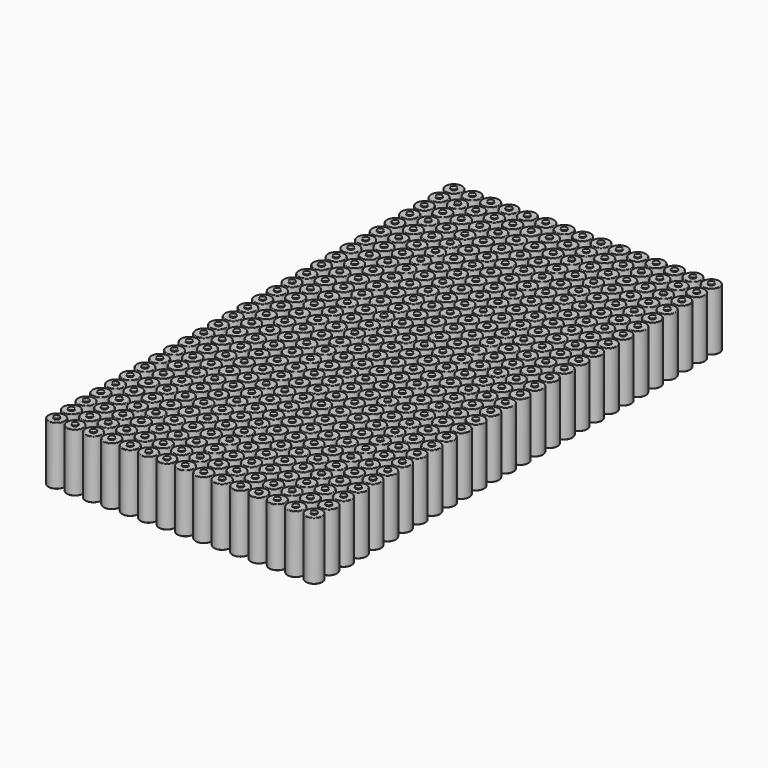
from build123d import *

# Parameters (mm, degrees)
F0_R      = 9.25
F1_DEPTH  = 32.5
F2_R      = 3.3
F3_DEPTH  = 1
F5_R      = 0.635
F6_R      = 0.635
F7_R      = 0.635
F8_R      = 0.635
F19_ANGLE = 90


with BuildPart() as f1:
    # F0 (on Top) → F1 (new body, symmetric)
    with BuildSketch(Plane.XY):
        Circle(F0_R)
    extrude(amount=F1_DEPTH, both=True)

    # F2 (on face) → F3 (join)
    with BuildSketch(Plane.XY.offset(32.5)):
        Circle(F2_R)
    extrude(amount=F3_DEPTH)


with BuildPart() as f4_1:
    # F4: copy of F1
    add(f1.part.moved(Location((20.5, 0, 0))))

    # F6
    f6_edges = [f4_1.edges().sort_by_distance(p)[0] for p in [
        (11.25, 0, 32.5),
    ]]
    fillet(f6_edges, radius=F6_R)

    # F8
    f8_edges = [f4_1.edges().sort_by_distance(p)[0] for p in [
        (11.25, 0, -32.5),
    ]]
    fillet(f8_edges, radius=F8_R)


with BuildPart() as f1_1:
    add(f1.part)

    # F5
    f5_edges = [f1_1.edges().sort_by_distance(p)[0] for p in [
        (-9.25, 0, 32.5),
    ]]
    fillet(f5_edges, radius=F5_R)

    # F7
    f7_edges = [f1_1.edges().sort_by_distance(p)[0] for p in [
        (-9.25, 0, -32.5),
        (9.25, 0, -0.3175),
        (-9.25, 0, 31.865),
    ]]
    fillet(f7_edges, radius=F7_R)


with BuildPart() as f9_1:
    # F9: copy of F1
    add(f1_1.part.moved(Location((-41, 0, 0))))


with BuildPart() as f9_2:
    # F9: copy of F4_1
    add(f4_1.part.moved(Location((-41, 0, 0))))


with BuildPart() as f10_1:
    # F10: copy of F1
    add(f1_1.part.moved(Location((41, 0, 0))))


with BuildPart() as f11_1:
    # F11: copy of F4_1
    add(f4_1.part.moved(Location((102.5, 0, 0))))


with BuildPart() as f11_2:
    # F11: copy of F1
    add(f1_1.part.moved(Location((102.5, 0, 0))))


with BuildPart() as f11_3:
    # F11: copy of F9_1
    add(f9_1.part.moved(Location((102.5, 0, 0))))


with BuildPart() as f11_4:
    # F11: copy of F10_1
    add(f10_1.part.moved(Location((102.5, 0, 0))))


with BuildPart() as f11_5:
    # F11: copy of F9_2
    add(f9_2.part.moved(Location((102.5, 0, 0))))


with BuildPart() as f12_1:
    # F12: copy of F1
    add(f1_1.part.moved(Location((-205, 0, 0))))


with BuildPart() as f12_2:
    # F12: copy of F4_1
    add(f4_1.part.moved(Location((-205, 0, 0))))


with BuildPart() as f12_3:
    # F12: copy of F9_1
    add(f9_1.part.moved(Location((-205, 0, 0))))


with BuildPart() as f12_4:
    # F12: copy of F10_1
    add(f10_1.part.moved(Location((-205, 0, 0))))


with BuildPart() as f12_5:
    # F12: copy of F11_3
    add(f11_3.part.moved(Location((-205, 0, 0))))


with BuildPart() as f12_6:
    # F12: copy of F11_4
    add(f11_4.part.moved(Location((-205, 0, 0))))


with BuildPart() as f12_7:
    # F12: copy of F11_5
    add(f11_5.part.moved(Location((-205, 0, 0))))


with BuildPart() as f12_8:
    # F12: copy of F11_1
    add(f11_1.part.moved(Location((-205, 0, 0))))


with BuildPart() as f12_9:
    # F12: copy of F11_2
    add(f11_2.part.moved(Location((-205, 0, 0))))


with BuildPart() as f12_10:
    # F12: copy of F9_2
    add(f9_2.part.moved(Location((-205, 0, 0))))


with BuildPart() as f1_2:
    # F13: moved
    add(f1_1.part.moved(Location((-30.75, 0, 0))))


with BuildPart() as f4_1_1:
    # F13: moved
    add(f4_1.part.moved(Location((-30.75, 0, 0))))


with BuildPart() as f9_2_1:
    # F13: moved
    add(f9_2.part.moved(Location((-30.75, 0, 0))))


with BuildPart() as f9_1_1:
    # F13: moved
    add(f9_1.part.moved(Location((-30.75, 0, 0))))


with BuildPart() as f10_1_1:
    # F13: moved
    add(f10_1.part.moved(Location((-30.75, 0, 0))))


with BuildPart() as f11_3_1:
    # F13: moved
    add(f11_3.part.moved(Location((-30.75, 0, 0))))


with BuildPart() as f11_4_1:
    # F13: moved
    add(f11_4.part.moved(Location((-30.75, 0, 0))))


with BuildPart() as f11_5_1:
    # F13: moved
    add(f11_5.part.moved(Location((-30.75, 0, 0))))


with BuildPart() as f11_1_1:
    # F13: moved
    add(f11_1.part.moved(Location((-30.75, 0, 0))))


with BuildPart() as f11_2_1:
    # F13: moved
    add(f11_2.part.moved(Location((-30.75, 0, 0))))


with BuildPart() as f12_8_1:
    # F13: moved
    add(f12_8.part.moved(Location((-30.75, 0, 0))))


with BuildPart() as f12_9_1:
    # F13: moved
    add(f12_9.part.moved(Location((-30.75, 0, 0))))


with BuildPart() as f12_7_1:
    # F13: moved
    add(f12_7.part.moved(Location((-30.75, 0, 0))))


with BuildPart() as f12_4_1:
    # F13: moved
    add(f12_4.part.moved(Location((-30.75, 0, 0))))


with BuildPart() as f12_10_1:
    # F13: moved
    add(f12_10.part.moved(Location((-30.75, 0, 0))))


with BuildPart() as f12_6_1:
    # F13: moved
    add(f12_6.part.moved(Location((-30.75, 0, 0))))


with BuildPart() as f12_5_1:
    # F13: moved
    add(f12_5.part.moved(Location((-30.75, 0, 0))))


with BuildPart() as f12_3_1:
    # F13: moved
    add(f12_3.part.moved(Location((-30.75, 0, 0))))


with BuildPart() as f12_2_1:
    # F13: moved
    add(f12_2.part.moved(Location((-30.75, 0, 0))))


with BuildPart() as f12_1_1:
    # F13: moved
    add(f12_1.part.moved(Location((-30.75, 0, 0))))


with BuildPart() as f14_1:
    # F14: copy of F4_1
    add(f4_1_1.part.moved(Location((164, 0, 0))))


with BuildPart() as f14_2:
    # F14: copy of F10_1
    add(f10_1_1.part.moved(Location((164, 0, 0))))


with BuildPart() as f14_3:
    # F14: copy of F11_3
    add(f11_3_1.part.moved(Location((164, 0, 0))))


with BuildPart() as f14_4:
    # F14: copy of F11_4
    add(f11_4_1.part.moved(Location((164, 0, 0))))


with BuildPart() as f14_5:
    # F14: copy of F11_5
    add(f11_5_1.part.moved(Location((164, 0, 0))))


with BuildPart() as f14_6:
    # F14: copy of F11_1
    add(f11_1_1.part.moved(Location((164, 0, 0))))


with BuildPart() as f14_7:
    # F14: copy of F11_2
    add(f11_2_1.part.moved(Location((164, 0, 0))))


with BuildPart() as f14_8:
    # F14: copy of F1
    add(f1_2.part.moved(Location((164, 0, 0))))


with BuildPart() as f15_1:
    # F15: copy of F4_1
    add(f4_1_1.part.moved(Location((0, -20.5, 0))))


with BuildPart() as f15_2:
    # F15: copy of F9_2
    add(f9_2_1.part.moved(Location((0, -20.5, 0))))


with BuildPart() as f15_3:
    # F15: copy of F9_1
    add(f9_1_1.part.moved(Location((0, -20.5, 0))))


with BuildPart() as f15_4:
    # F15: copy of F10_1
    add(f10_1_1.part.moved(Location((0, -20.5, 0))))


with BuildPart() as f15_5:
    # F15: copy of F11_3
    add(f11_3_1.part.moved(Location((0, -20.5, 0))))


with BuildPart() as f15_6:
    # F15: copy of F11_4
    add(f11_4_1.part.moved(Location((0, -20.5, 0))))


with BuildPart() as f15_7:
    # F15: copy of F11_5
    add(f11_5_1.part.moved(Location((0, -20.5, 0))))


with BuildPart() as f15_8:
    # F15: copy of F11_1
    add(f11_1_1.part.moved(Location((0, -20.5, 0))))


with BuildPart() as f15_9:
    # F15: copy of F11_2
    add(f11_2_1.part.moved(Location((0, -20.5, 0))))


with BuildPart() as f15_10:
    # F15: copy of F12_9
    add(f12_9_1.part.moved(Location((0, -20.5, 0))))


with BuildPart() as f15_11:
    # F15: copy of F12_7
    add(f12_7_1.part.moved(Location((0, -20.5, 0))))


with BuildPart() as f15_12:
    # F15: copy of F12_4
    add(f12_4_1.part.moved(Location((0, -20.5, 0))))


with BuildPart() as f15_13:
    # F15: copy of F12_10
    add(f12_10_1.part.moved(Location((0, -20.5, 0))))


with BuildPart() as f15_14:
    # F15: copy of F12_8
    add(f12_8_1.part.moved(Location((0, -20.5, 0))))


with BuildPart() as f15_15:
    # F15: copy of F12_6
    add(f12_6_1.part.moved(Location((0, -20.5, 0))))


with BuildPart() as f15_16:
    # F15: copy of F12_3
    add(f12_3_1.part.moved(Location((0, -20.5, 0))))


with BuildPart() as f15_17:
    # F15: copy of F12_5
    add(f12_5_1.part.moved(Location((0, -20.5, 0))))


with BuildPart() as f15_18:
    # F15: copy of F12_2
    add(f12_2_1.part.moved(Location((0, -20.5, 0))))


with BuildPart() as f15_19:
    # F15: copy of F12_1
    add(f12_1_1.part.moved(Location((0, -20.5, 0))))


with BuildPart() as f15_20:
    # F15: copy of F14_4
    add(f14_4.part.moved(Location((0, -20.5, 0))))


with BuildPart() as f15_21:
    # F15: copy of F14_5
    add(f14_5.part.moved(Location((0, -20.5, 0))))


with BuildPart() as f15_22:
    # F15: copy of F14_7
    add(f14_7.part.moved(Location((0, -20.5, 0))))


with BuildPart() as f15_23:
    # F15: copy of F14_3
    add(f14_3.part.moved(Location((0, -20.5, 0))))


with BuildPart() as f15_24:
    # F15: copy of F14_6
    add(f14_6.part.moved(Location((0, -20.5, 0))))


with BuildPart() as f15_25:
    # F15: copy of F14_2
    add(f14_2.part.moved(Location((0, -20.5, 0))))


with BuildPart() as f15_26:
    # F15: copy of F14_1
    add(f14_1.part.moved(Location((0, -20.5, 0))))


with BuildPart() as f15_27:
    # F15: copy of F14_8
    add(f14_8.part.moved(Location((0, -20.5, 0))))


with BuildPart() as f15_28:
    # F15: copy of F1
    add(f1_2.part.moved(Location((0, -20.5, 0))))


with BuildPart() as f16_1:
    # F16: copy of F4_1
    add(f4_1_1.part.moved(Location((0, -41, 0))))


with BuildPart() as f16_2:
    # F16: copy of F9_2
    add(f9_2_1.part.moved(Location((0, -41, 0))))


with BuildPart() as f16_3:
    # F16: copy of F9_1
    add(f9_1_1.part.moved(Location((0, -41, 0))))


with BuildPart() as f16_4:
    # F16: copy of F10_1
    add(f10_1_1.part.moved(Location((0, -41, 0))))


with BuildPart() as f16_5:
    # F16: copy of F11_3
    add(f11_3_1.part.moved(Location((0, -41, 0))))


with BuildPart() as f16_6:
    # F16: copy of F11_4
    add(f11_4_1.part.moved(Location((0, -41, 0))))


with BuildPart() as f16_7:
    # F16: copy of F11_1
    add(f11_1_1.part.moved(Location((0, -41, 0))))


with BuildPart() as f16_8:
    # F16: copy of F11_5
    add(f11_5_1.part.moved(Location((0, -41, 0))))


with BuildPart() as f16_9:
    # F16: copy of F11_2
    add(f11_2_1.part.moved(Location((0, -41, 0))))


with BuildPart() as f16_10:
    # F16: copy of F12_3
    add(f12_3_1.part.moved(Location((0, -41, 0))))


with BuildPart() as f16_11:
    # F16: copy of F12_9
    add(f12_9_1.part.moved(Location((0, -41, 0))))


with BuildPart() as f16_12:
    # F16: copy of F12_7
    add(f12_7_1.part.moved(Location((0, -41, 0))))


with BuildPart() as f16_13:
    # F16: copy of F12_4
    add(f12_4_1.part.moved(Location((0, -41, 0))))


with BuildPart() as f16_14:
    # F16: copy of F12_10
    add(f12_10_1.part.moved(Location((0, -41, 0))))


with BuildPart() as f16_15:
    # F16: copy of F12_6
    add(f12_6_1.part.moved(Location((0, -41, 0))))


with BuildPart() as f16_16:
    # F16: copy of F12_8
    add(f12_8_1.part.moved(Location((0, -41, 0))))


with BuildPart() as f16_17:
    # F16: copy of F12_2
    add(f12_2_1.part.moved(Location((0, -41, 0))))


with BuildPart() as f16_18:
    # F16: copy of F12_1
    add(f12_1_1.part.moved(Location((0, -41, 0))))


with BuildPart() as f16_19:
    # F16: copy of F12_5
    add(f12_5_1.part.moved(Location((0, -41, 0))))


with BuildPart() as f16_20:
    # F16: copy of F14_4
    add(f14_4.part.moved(Location((0, -41, 0))))


with BuildPart() as f16_21:
    # F16: copy of F14_7
    add(f14_7.part.moved(Location((0, -41, 0))))


with BuildPart() as f16_22:
    # F16: copy of F14_5
    add(f14_5.part.moved(Location((0, -41, 0))))


with BuildPart() as f16_23:
    # F16: copy of F14_3
    add(f14_3.part.moved(Location((0, -41, 0))))


with BuildPart() as f16_24:
    # F16: copy of F14_6
    add(f14_6.part.moved(Location((0, -41, 0))))


with BuildPart() as f16_25:
    # F16: copy of F14_2
    add(f14_2.part.moved(Location((0, -41, 0))))


with BuildPart() as f16_26:
    # F16: copy of F14_1
    add(f14_1.part.moved(Location((0, -41, 0))))


with BuildPart() as f16_27:
    # F16: copy of F14_8
    add(f14_8.part.moved(Location((0, -41, 0))))


with BuildPart() as f16_28:
    # F16: copy of F15_11
    add(f15_11.part.moved(Location((0, -41, 0))))


with BuildPart() as f16_29:
    # F16: copy of F15_25
    add(f15_25.part.moved(Location((0, -41, 0))))


with BuildPart() as f16_30:
    # F16: copy of F15_10
    add(f15_10.part.moved(Location((0, -41, 0))))


with BuildPart() as f16_31:
    # F16: copy of F15_22
    add(f15_22.part.moved(Location((0, -41, 0))))


with BuildPart() as f16_32:
    # F16: copy of F15_19
    add(f15_19.part.moved(Location((0, -41, 0))))


with BuildPart() as f16_33:
    # F16: copy of F15_13
    add(f15_13.part.moved(Location((0, -41, 0))))


with BuildPart() as f16_34:
    # F16: copy of F15_21
    add(f15_21.part.moved(Location((0, -41, 0))))


with BuildPart() as f16_35:
    # F16: copy of F15_6
    add(f15_6.part.moved(Location((0, -41, 0))))


with BuildPart() as f16_36:
    # F16: copy of F15_7
    add(f15_7.part.moved(Location((0, -41, 0))))


with BuildPart() as f16_37:
    # F16: copy of F15_9
    add(f15_9.part.moved(Location((0, -41, 0))))


with BuildPart() as f16_38:
    # F16: copy of F15_3
    add(f15_3.part.moved(Location((0, -41, 0))))


with BuildPart() as f16_39:
    # F16: copy of F15_23
    add(f15_23.part.moved(Location((0, -41, 0))))


with BuildPart() as f16_40:
    # F16: copy of F15_26
    add(f15_26.part.moved(Location((0, -41, 0))))


with BuildPart() as f16_41:
    # F16: copy of F15_12
    add(f15_12.part.moved(Location((0, -41, 0))))


with BuildPart() as f16_42:
    # F16: copy of F15_18
    add(f15_18.part.moved(Location((0, -41, 0))))


with BuildPart() as f16_43:
    # F16: copy of F15_20
    add(f15_20.part.moved(Location((0, -41, 0))))


with BuildPart() as f16_44:
    # F16: copy of F15_24
    add(f15_24.part.moved(Location((0, -41, 0))))


with BuildPart() as f16_45:
    # F16: copy of F15_8
    add(f15_8.part.moved(Location((0, -41, 0))))


with BuildPart() as f16_46:
    # F16: copy of F15_4
    add(f15_4.part.moved(Location((0, -41, 0))))


with BuildPart() as f16_47:
    # F16: copy of F15_2
    add(f15_2.part.moved(Location((0, -41, 0))))


with BuildPart() as f16_48:
    # F16: copy of F15_15
    add(f15_15.part.moved(Location((0, -41, 0))))


with BuildPart() as f16_49:
    # F16: copy of F15_17
    add(f15_17.part.moved(Location((0, -41, 0))))


with BuildPart() as f16_50:
    # F16: copy of F15_14
    add(f15_14.part.moved(Location((0, -41, 0))))


with BuildPart() as f16_51:
    # F16: copy of F15_16
    add(f15_16.part.moved(Location((0, -41, 0))))


with BuildPart() as f16_52:
    # F16: copy of F15_1
    add(f15_1.part.moved(Location((0, -41, 0))))


with BuildPart() as f16_53:
    # F16: copy of F15_27
    add(f15_27.part.moved(Location((0, -41, 0))))


with BuildPart() as f16_54:
    # F16: copy of F15_5
    add(f15_5.part.moved(Location((0, -41, 0))))


with BuildPart() as f16_55:
    # F16: copy of F15_28
    add(f15_28.part.moved(Location((0, -41, 0))))


with BuildPart() as f16_56:
    # F16: copy of F1
    add(f1_2.part.moved(Location((0, -41, 0))))


with BuildPart() as f17_1:
    # F17: copy of F4_1
    add(f4_1_1.part.moved(Location((0, -82, 0))))


with BuildPart() as f17_2:
    # F17: copy of F9_2
    add(f9_2_1.part.moved(Location((0, -82, 0))))


with BuildPart() as f17_3:
    # F17: copy of F9_1
    add(f9_1_1.part.moved(Location((0, -82, 0))))


with BuildPart() as f17_4:
    # F17: copy of F10_1
    add(f10_1_1.part.moved(Location((0, -82, 0))))


with BuildPart() as f17_5:
    # F17: copy of F11_4
    add(f11_4_1.part.moved(Location((0, -82, 0))))


with BuildPart() as f17_6:
    # F17: copy of F11_3
    add(f11_3_1.part.moved(Location((0, -82, 0))))


with BuildPart() as f17_7:
    # F17: copy of F11_5
    add(f11_5_1.part.moved(Location((0, -82, 0))))


with BuildPart() as f17_8:
    # F17: copy of F11_1
    add(f11_1_1.part.moved(Location((0, -82, 0))))


with BuildPart() as f17_9:
    # F17: copy of F11_2
    add(f11_2_1.part.moved(Location((0, -82, 0))))


with BuildPart() as f17_10:
    # F17: copy of F12_9
    add(f12_9_1.part.moved(Location((0, -82, 0))))


with BuildPart() as f17_11:
    # F17: copy of F12_7
    add(f12_7_1.part.moved(Location((0, -82, 0))))


with BuildPart() as f17_12:
    # F17: copy of F12_4
    add(f12_4_1.part.moved(Location((0, -82, 0))))


with BuildPart() as f17_13:
    # F17: copy of F12_6
    add(f12_6_1.part.moved(Location((0, -82, 0))))


with BuildPart() as f17_14:
    # F17: copy of F12_3
    add(f12_3_1.part.moved(Location((0, -82, 0))))


with BuildPart() as f17_15:
    # F17: copy of F12_8
    add(f12_8_1.part.moved(Location((0, -82, 0))))


with BuildPart() as f17_16:
    # F17: copy of F12_2
    add(f12_2_1.part.moved(Location((0, -82, 0))))


with BuildPart() as f17_17:
    # F17: copy of F12_1
    add(f12_1_1.part.moved(Location((0, -82, 0))))


with BuildPart() as f17_18:
    # F17: copy of F12_10
    add(f12_10_1.part.moved(Location((0, -82, 0))))


with BuildPart() as f17_19:
    # F17: copy of F12_5
    add(f12_5_1.part.moved(Location((0, -82, 0))))


with BuildPart() as f17_20:
    # F17: copy of F14_4
    add(f14_4.part.moved(Location((0, -82, 0))))


with BuildPart() as f17_21:
    # F17: copy of F14_7
    add(f14_7.part.moved(Location((0, -82, 0))))


with BuildPart() as f17_22:
    # F17: copy of F14_5
    add(f14_5.part.moved(Location((0, -82, 0))))


with BuildPart() as f17_23:
    # F17: copy of F14_3
    add(f14_3.part.moved(Location((0, -82, 0))))


with BuildPart() as f17_24:
    # F17: copy of F14_6
    add(f14_6.part.moved(Location((0, -82, 0))))


with BuildPart() as f17_25:
    # F17: copy of F14_2
    add(f14_2.part.moved(Location((0, -82, 0))))


with BuildPart() as f17_26:
    # F17: copy of F14_1
    add(f14_1.part.moved(Location((0, -82, 0))))


with BuildPart() as f17_27:
    # F17: copy of F14_8
    add(f14_8.part.moved(Location((0, -82, 0))))


with BuildPart() as f17_28:
    # F17: copy of F15_11
    add(f15_11.part.moved(Location((0, -82, 0))))


with BuildPart() as f17_29:
    # F17: copy of F15_25
    add(f15_25.part.moved(Location((0, -82, 0))))


with BuildPart() as f17_30:
    # F17: copy of F15_10
    add(f15_10.part.moved(Location((0, -82, 0))))


with BuildPart() as f17_31:
    # F17: copy of F15_19
    add(f15_19.part.moved(Location((0, -82, 0))))


with BuildPart() as f17_32:
    # F17: copy of F15_13
    add(f15_13.part.moved(Location((0, -82, 0))))


with BuildPart() as f17_33:
    # F17: copy of F15_7
    add(f15_7.part.moved(Location((0, -82, 0))))


with BuildPart() as f17_34:
    # F17: copy of F15_9
    add(f15_9.part.moved(Location((0, -82, 0))))


with BuildPart() as f17_35:
    # F17: copy of F15_3
    add(f15_3.part.moved(Location((0, -82, 0))))


with BuildPart() as f17_36:
    # F17: copy of F15_12
    add(f15_12.part.moved(Location((0, -82, 0))))


with BuildPart() as f17_37:
    # F17: copy of F15_18
    add(f15_18.part.moved(Location((0, -82, 0))))


with BuildPart() as f17_38:
    # F17: copy of F15_20
    add(f15_20.part.moved(Location((0, -82, 0))))


with BuildPart() as f17_39:
    # F17: copy of F15_24
    add(f15_24.part.moved(Location((0, -82, 0))))


with BuildPart() as f17_40:
    # F17: copy of F15_26
    add(f15_26.part.moved(Location((0, -82, 0))))


with BuildPart() as f17_41:
    # F17: copy of F15_8
    add(f15_8.part.moved(Location((0, -82, 0))))


with BuildPart() as f17_42:
    # F17: copy of F15_2
    add(f15_2.part.moved(Location((0, -82, 0))))


with BuildPart() as f17_43:
    # F17: copy of F15_22
    add(f15_22.part.moved(Location((0, -82, 0))))


with BuildPart() as f17_44:
    # F17: copy of F15_15
    add(f15_15.part.moved(Location((0, -82, 0))))


with BuildPart() as f17_45:
    # F17: copy of F15_17
    add(f15_17.part.moved(Location((0, -82, 0))))


with BuildPart() as f17_46:
    # F17: copy of F15_23
    add(f15_23.part.moved(Location((0, -82, 0))))


with BuildPart() as f17_47:
    # F17: copy of F15_16
    add(f15_16.part.moved(Location((0, -82, 0))))


with BuildPart() as f17_48:
    # F17: copy of F15_14
    add(f15_14.part.moved(Location((0, -82, 0))))


with BuildPart() as f17_49:
    # F17: copy of F15_28
    add(f15_28.part.moved(Location((0, -82, 0))))


with BuildPart() as f17_50:
    # F17: copy of F15_1
    add(f15_1.part.moved(Location((0, -82, 0))))


with BuildPart() as f17_51:
    # F17: copy of F15_6
    add(f15_6.part.moved(Location((0, -82, 0))))


with BuildPart() as f17_52:
    # F17: copy of F15_5
    add(f15_5.part.moved(Location((0, -82, 0))))


with BuildPart() as f17_53:
    # F17: copy of F15_4
    add(f15_4.part.moved(Location((0, -82, 0))))


with BuildPart() as f17_54:
    # F17: copy of F15_21
    add(f15_21.part.moved(Location((0, -82, 0))))


with BuildPart() as f17_55:
    # F17: copy of F15_27
    add(f15_27.part.moved(Location((0, -82, 0))))


with BuildPart() as f17_56:
    # F17: copy of F16_10
    add(f16_10.part.moved(Location((0, -82, 0))))


with BuildPart() as f17_57:
    # F17: copy of F16_13
    add(f16_13.part.moved(Location((0, -82, 0))))


with BuildPart() as f17_58:
    # F17: copy of F16_2
    add(f16_2.part.moved(Location((0, -82, 0))))


with BuildPart() as f17_59:
    # F17: copy of F16_9
    add(f16_9.part.moved(Location((0, -82, 0))))


with BuildPart() as f17_60:
    # F17: copy of F16_23
    add(f16_23.part.moved(Location((0, -82, 0))))


with BuildPart() as f17_61:
    # F17: copy of F16_24
    add(f16_24.part.moved(Location((0, -82, 0))))


with BuildPart() as f17_62:
    # F17: copy of F16_12
    add(f16_12.part.moved(Location((0, -82, 0))))


with BuildPart() as f17_63:
    # F17: copy of F16_45
    add(f16_45.part.moved(Location((0, -82, 0))))


with BuildPart() as f17_64:
    # F17: copy of F16_47
    add(f16_47.part.moved(Location((0, -82, 0))))


with BuildPart() as f17_65:
    # F17: copy of F16_55
    add(f16_55.part.moved(Location((0, -82, 0))))


with BuildPart() as f17_66:
    # F17: copy of F16_50
    add(f16_50.part.moved(Location((0, -82, 0))))


with BuildPart() as f17_67:
    # F17: copy of F16_32
    add(f16_32.part.moved(Location((0, -82, 0))))


with BuildPart() as f17_68:
    # F17: copy of F16_35
    add(f16_35.part.moved(Location((0, -82, 0))))


with BuildPart() as f17_69:
    # F17: copy of F16_39
    add(f16_39.part.moved(Location((0, -82, 0))))


with BuildPart() as f17_70:
    # F17: copy of F16_29
    add(f16_29.part.moved(Location((0, -82, 0))))


with BuildPart() as f17_71:
    # F17: copy of F16_53
    add(f16_53.part.moved(Location((0, -82, 0))))


with BuildPart() as f17_72:
    # F17: copy of F16_43
    add(f16_43.part.moved(Location((0, -82, 0))))


with BuildPart() as f17_73:
    # F17: copy of F16_20
    add(f16_20.part.moved(Location((0, -82, 0))))


with BuildPart() as f17_74:
    # F17: copy of F16_7
    add(f16_7.part.moved(Location((0, -82, 0))))


with BuildPart() as f17_75:
    # F17: copy of F16_6
    add(f16_6.part.moved(Location((0, -82, 0))))


with BuildPart() as f17_76:
    # F17: copy of F16_1
    add(f16_1.part.moved(Location((0, -82, 0))))


with BuildPart() as f17_77:
    # F17: copy of F16_3
    add(f16_3.part.moved(Location((0, -82, 0))))


with BuildPart() as f17_78:
    # F17: copy of F16_56
    add(f16_56.part.moved(Location((0, -82, 0))))


with BuildPart() as f17_79:
    # F17: copy of F16_15
    add(f16_15.part.moved(Location((0, -82, 0))))


with BuildPart() as f17_80:
    # F17: copy of F16_30
    add(f16_30.part.moved(Location((0, -82, 0))))


with BuildPart() as f17_81:
    # F17: copy of F16_33
    add(f16_33.part.moved(Location((0, -82, 0))))


with BuildPart() as f17_82:
    # F17: copy of F16_42
    add(f16_42.part.moved(Location((0, -82, 0))))


with BuildPart() as f17_83:
    # F17: copy of F16_34
    add(f16_34.part.moved(Location((0, -82, 0))))


with BuildPart() as f17_84:
    # F17: copy of F16_31
    add(f16_31.part.moved(Location((0, -82, 0))))


with BuildPart() as f17_85:
    # F17: copy of F16_49
    add(f16_49.part.moved(Location((0, -82, 0))))


with BuildPart() as f17_86:
    # F17: copy of F16_14
    add(f16_14.part.moved(Location((0, -82, 0))))


with BuildPart() as f17_87:
    # F17: copy of F16_27
    add(f16_27.part.moved(Location((0, -82, 0))))


with BuildPart() as f17_88:
    # F17: copy of F16_16
    add(f16_16.part.moved(Location((0, -82, 0))))


with BuildPart() as f17_89:
    # F17: copy of F16_38
    add(f16_38.part.moved(Location((0, -82, 0))))


with BuildPart() as f17_90:
    # F17: copy of F16_52
    add(f16_52.part.moved(Location((0, -82, 0))))


with BuildPart() as f17_91:
    # F17: copy of F16_22
    add(f16_22.part.moved(Location((0, -82, 0))))


with BuildPart() as f17_92:
    # F17: copy of F16_21
    add(f16_21.part.moved(Location((0, -82, 0))))


with BuildPart() as f17_93:
    # F17: copy of F16_46
    add(f16_46.part.moved(Location((0, -82, 0))))


with BuildPart() as f17_94:
    # F17: copy of F16_40
    add(f16_40.part.moved(Location((0, -82, 0))))


with BuildPart() as f17_95:
    # F17: copy of F16_28
    add(f16_28.part.moved(Location((0, -82, 0))))


with BuildPart() as f17_96:
    # F17: copy of F16_41
    add(f16_41.part.moved(Location((0, -82, 0))))


with BuildPart() as f17_97:
    # F17: copy of F16_18
    add(f16_18.part.moved(Location((0, -82, 0))))


with BuildPart() as f17_98:
    # F17: copy of F16_8
    add(f16_8.part.moved(Location((0, -82, 0))))


with BuildPart() as f17_99:
    # F17: copy of F16_19
    add(f16_19.part.moved(Location((0, -82, 0))))


with BuildPart() as f17_100:
    # F17: copy of F16_37
    add(f16_37.part.moved(Location((0, -82, 0))))


with BuildPart() as f17_101:
    # F17: copy of F16_17
    add(f16_17.part.moved(Location((0, -82, 0))))


with BuildPart() as f17_102:
    # F17: copy of F16_51
    add(f16_51.part.moved(Location((0, -82, 0))))


with BuildPart() as f17_103:
    # F17: copy of F16_44
    add(f16_44.part.moved(Location((0, -82, 0))))


with BuildPart() as f17_104:
    # F17: copy of F16_26
    add(f16_26.part.moved(Location((0, -82, 0))))


with BuildPart() as f17_105:
    # F17: copy of F16_11
    add(f16_11.part.moved(Location((0, -82, 0))))


with BuildPart() as f17_106:
    # F17: copy of F16_54
    add(f16_54.part.moved(Location((0, -82, 0))))


with BuildPart() as f17_107:
    # F17: copy of F16_48
    add(f16_48.part.moved(Location((0, -82, 0))))


with BuildPart() as f17_108:
    # F17: copy of F16_25
    add(f16_25.part.moved(Location((0, -82, 0))))


with BuildPart() as f17_109:
    # F17: copy of F16_36
    add(f16_36.part.moved(Location((0, -82, 0))))


with BuildPart() as f17_110:
    # F17: copy of F16_4
    add(f16_4.part.moved(Location((0, -82, 0))))


with BuildPart() as f17_111:
    # F17: copy of F1
    add(f1_2.part.moved(Location((0, -82, 0))))


with BuildPart() as f17_112:
    # F17: copy of F16_5
    add(f16_5.part.moved(Location((0, -82, 0))))


with BuildPart() as f18_1:
    # F18: copy of F1
    add(f1_2.part.moved(Location((0, 143.5, 0))))


with BuildPart() as f18_2:
    # F18: copy of F4_1
    add(f4_1_1.part.moved(Location((0, 143.5, 0))))


with BuildPart() as f18_3:
    # F18: copy of F9_2
    add(f9_2_1.part.moved(Location((0, 143.5, 0))))


with BuildPart() as f18_4:
    # F18: copy of F9_1
    add(f9_1_1.part.moved(Location((0, 143.5, 0))))


with BuildPart() as f18_5:
    # F18: copy of F10_1
    add(f10_1_1.part.moved(Location((0, 143.5, 0))))


with BuildPart() as f18_6:
    # F18: copy of F11_4
    add(f11_4_1.part.moved(Location((0, 143.5, 0))))


with BuildPart() as f18_7:
    # F18: copy of F11_3
    add(f11_3_1.part.moved(Location((0, 143.5, 0))))


with BuildPart() as f18_8:
    # F18: copy of F11_5
    add(f11_5_1.part.moved(Location((0, 143.5, 0))))


with BuildPart() as f18_9:
    # F18: copy of F11_2
    add(f11_2_1.part.moved(Location((0, 143.5, 0))))


with BuildPart() as f18_10:
    # F18: copy of F11_1
    add(f11_1_1.part.moved(Location((0, 143.5, 0))))


with BuildPart() as f18_11:
    # F18: copy of F12_3
    add(f12_3_1.part.moved(Location((0, 143.5, 0))))


with BuildPart() as f18_12:
    # F18: copy of F12_10
    add(f12_10_1.part.moved(Location((0, 143.5, 0))))


with BuildPart() as f18_13:
    # F18: copy of F12_9
    add(f12_9_1.part.moved(Location((0, 143.5, 0))))


with BuildPart() as f18_14:
    # F18: copy of F12_7
    add(f12_7_1.part.moved(Location((0, 143.5, 0))))


with BuildPart() as f18_15:
    # F18: copy of F12_4
    add(f12_4_1.part.moved(Location((0, 143.5, 0))))


with BuildPart() as f18_16:
    # F18: copy of F12_5
    add(f12_5_1.part.moved(Location((0, 143.5, 0))))


with BuildPart() as f18_17:
    # F18: copy of F12_8
    add(f12_8_1.part.moved(Location((0, 143.5, 0))))


with BuildPart() as f18_18:
    # F18: copy of F12_6
    add(f12_6_1.part.moved(Location((0, 143.5, 0))))


with BuildPart() as f18_19:
    # F18: copy of F12_1
    add(f12_1_1.part.moved(Location((0, 143.5, 0))))


with BuildPart() as f18_20:
    # F18: copy of F12_2
    add(f12_2_1.part.moved(Location((0, 143.5, 0))))


with BuildPart() as f18_21:
    # F18: copy of F14_7
    add(f14_7.part.moved(Location((0, 143.5, 0))))


with BuildPart() as f18_22:
    # F18: copy of F14_4
    add(f14_4.part.moved(Location((0, 143.5, 0))))


with BuildPart() as f18_23:
    # F18: copy of F14_3
    add(f14_3.part.moved(Location((0, 143.5, 0))))


with BuildPart() as f18_24:
    # F18: copy of F14_5
    add(f14_5.part.moved(Location((0, 143.5, 0))))


with BuildPart() as f18_25:
    # F18: copy of F14_6
    add(f14_6.part.moved(Location((0, 143.5, 0))))


with BuildPart() as f18_26:
    # F18: copy of F14_2
    add(f14_2.part.moved(Location((0, 143.5, 0))))


with BuildPart() as f18_27:
    # F18: copy of F14_8
    add(f14_8.part.moved(Location((0, 143.5, 0))))


with BuildPart() as f18_28:
    # F18: copy of F14_1
    add(f14_1.part.moved(Location((0, 143.5, 0))))


with BuildPart() as f18_29:
    # F18: copy of F15_11
    add(f15_11.part.moved(Location((0, 143.5, 0))))


with BuildPart() as f18_30:
    # F18: copy of F15_10
    add(f15_10.part.moved(Location((0, 143.5, 0))))


with BuildPart() as f18_31:
    # F18: copy of F15_19
    add(f15_19.part.moved(Location((0, 143.5, 0))))


with BuildPart() as f18_32:
    # F18: copy of F15_13
    add(f15_13.part.moved(Location((0, 143.5, 0))))


with BuildPart() as f18_33:
    # F18: copy of F15_5
    add(f15_5.part.moved(Location((0, 143.5, 0))))


with BuildPart() as f18_34:
    # F18: copy of F15_3
    add(f15_3.part.moved(Location((0, 143.5, 0))))


with BuildPart() as f18_35:
    # F18: copy of F15_12
    add(f15_12.part.moved(Location((0, 143.5, 0))))


with BuildPart() as f18_36:
    # F18: copy of F15_17
    add(f15_17.part.moved(Location((0, 143.5, 0))))


with BuildPart() as f18_37:
    # F18: copy of F15_20
    add(f15_20.part.moved(Location((0, 143.5, 0))))


with BuildPart() as f18_38:
    # F18: copy of F15_23
    add(f15_23.part.moved(Location((0, 143.5, 0))))


with BuildPart() as f18_39:
    # F18: copy of F15_26
    add(f15_26.part.moved(Location((0, 143.5, 0))))


with BuildPart() as f18_40:
    # F18: copy of F15_8
    add(f15_8.part.moved(Location((0, 143.5, 0))))


with BuildPart() as f18_41:
    # F18: copy of F15_21
    add(f15_21.part.moved(Location((0, 143.5, 0))))


with BuildPart() as f18_42:
    # F18: copy of F15_27
    add(f15_27.part.moved(Location((0, 143.5, 0))))


with BuildPart() as f18_43:
    # F18: copy of F15_7
    add(f15_7.part.moved(Location((0, 143.5, 0))))


with BuildPart() as f18_44:
    # F18: copy of F15_4
    add(f15_4.part.moved(Location((0, 143.5, 0))))


with BuildPart() as f18_45:
    # F18: copy of F15_9
    add(f15_9.part.moved(Location((0, 143.5, 0))))


with BuildPart() as f18_46:
    # F18: copy of F15_2
    add(f15_2.part.moved(Location((0, 143.5, 0))))


with BuildPart() as f18_47:
    # F18: copy of F15_25
    add(f15_25.part.moved(Location((0, 143.5, 0))))


with BuildPart() as f18_48:
    # F18: copy of F15_18
    add(f15_18.part.moved(Location((0, 143.5, 0))))


with BuildPart() as f18_49:
    # F18: copy of F15_24
    add(f15_24.part.moved(Location((0, 143.5, 0))))


with BuildPart() as f18_50:
    # F18: copy of F15_28
    add(f15_28.part.moved(Location((0, 143.5, 0))))


with BuildPart() as f18_51:
    # F18: copy of F15_1
    add(f15_1.part.moved(Location((0, 143.5, 0))))


with BuildPart() as f18_52:
    # F18: copy of F15_16
    add(f15_16.part.moved(Location((0, 143.5, 0))))


with BuildPart() as f18_53:
    # F18: copy of F15_15
    add(f15_15.part.moved(Location((0, 143.5, 0))))


with BuildPart() as f18_54:
    # F18: copy of F15_22
    add(f15_22.part.moved(Location((0, 143.5, 0))))


with BuildPart() as f18_55:
    # F18: copy of F15_14
    add(f15_14.part.moved(Location((0, 143.5, 0))))


with BuildPart() as f18_56:
    # F18: copy of F15_6
    add(f15_6.part.moved(Location((0, 143.5, 0))))


with BuildPart() as f18_57:
    # F18: copy of F16_10
    add(f16_10.part.moved(Location((0, 143.5, 0))))


with BuildPart() as f18_58:
    # F18: copy of F16_13
    add(f16_13.part.moved(Location((0, 143.5, 0))))


with BuildPart() as f18_59:
    # F18: copy of F16_7
    add(f16_7.part.moved(Location((0, 143.5, 0))))


with BuildPart() as f18_60:
    # F18: copy of F16_2
    add(f16_2.part.moved(Location((0, 143.5, 0))))


with BuildPart() as f18_61:
    # F18: copy of F16_9
    add(f16_9.part.moved(Location((0, 143.5, 0))))


with BuildPart() as f18_62:
    # F18: copy of F16_8
    add(f16_8.part.moved(Location((0, 143.5, 0))))


with BuildPart() as f18_63:
    # F18: copy of F16_51
    add(f16_51.part.moved(Location((0, 143.5, 0))))


with BuildPart() as f18_64:
    # F18: copy of F16_23
    add(f16_23.part.moved(Location((0, 143.5, 0))))


with BuildPart() as f18_65:
    # F18: copy of F16_53
    add(f16_53.part.moved(Location((0, 143.5, 0))))


with BuildPart() as f18_66:
    # F18: copy of F16_32
    add(f16_32.part.moved(Location((0, 143.5, 0))))


with BuildPart() as f18_67:
    # F18: copy of F16_24
    add(f16_24.part.moved(Location((0, 143.5, 0))))


with BuildPart() as f18_68:
    # F18: copy of F16_45
    add(f16_45.part.moved(Location((0, 143.5, 0))))


with BuildPart() as f18_69:
    # F18: copy of F16_47
    add(f16_47.part.moved(Location((0, 143.5, 0))))


with BuildPart() as f18_70:
    # F18: copy of F16_50
    add(f16_50.part.moved(Location((0, 143.5, 0))))


with BuildPart() as f18_71:
    # F18: copy of F16_35
    add(f16_35.part.moved(Location((0, 143.5, 0))))


with BuildPart() as f18_72:
    # F18: copy of F16_39
    add(f16_39.part.moved(Location((0, 143.5, 0))))


with BuildPart() as f18_73:
    # F18: copy of F16_43
    add(f16_43.part.moved(Location((0, 143.5, 0))))


with BuildPart() as f18_74:
    # F18: copy of F16_20
    add(f16_20.part.moved(Location((0, 143.5, 0))))


with BuildPart() as f18_75:
    # F18: copy of F16_15
    add(f16_15.part.moved(Location((0, 143.5, 0))))


with BuildPart() as f18_76:
    # F18: copy of F16_28
    add(f16_28.part.moved(Location((0, 143.5, 0))))


with BuildPart() as f18_77:
    # F18: copy of F16_34
    add(f16_34.part.moved(Location((0, 143.5, 0))))


with BuildPart() as f18_78:
    # F18: copy of F16_5
    add(f16_5.part.moved(Location((0, 143.5, 0))))


with BuildPart() as f18_79:
    # F18: copy of F16_3
    add(f16_3.part.moved(Location((0, 143.5, 0))))


with BuildPart() as f18_80:
    # F18: copy of F16_56
    add(f16_56.part.moved(Location((0, 143.5, 0))))


with BuildPart() as f18_81:
    # F18: copy of F16_22
    add(f16_22.part.moved(Location((0, 143.5, 0))))


with BuildPart() as f18_82:
    # F18: copy of F16_21
    add(f16_21.part.moved(Location((0, 143.5, 0))))


with BuildPart() as f18_83:
    # F18: copy of F16_1
    add(f16_1.part.moved(Location((0, 143.5, 0))))


with BuildPart() as f18_84:
    # F18: copy of F16_55
    add(f16_55.part.moved(Location((0, 143.5, 0))))


with BuildPart() as f18_85:
    # F18: copy of F16_33
    add(f16_33.part.moved(Location((0, 143.5, 0))))


with BuildPart() as f18_86:
    # F18: copy of F16_54
    add(f16_54.part.moved(Location((0, 143.5, 0))))


with BuildPart() as f18_87:
    # F18: copy of F16_40
    add(f16_40.part.moved(Location((0, 143.5, 0))))


with BuildPart() as f18_88:
    # F18: copy of F16_14
    add(f16_14.part.moved(Location((0, 143.5, 0))))


with BuildPart() as f18_89:
    # F18: copy of F16_38
    add(f16_38.part.moved(Location((0, 143.5, 0))))


with BuildPart() as f18_90:
    # F18: copy of F16_31
    add(f16_31.part.moved(Location((0, 143.5, 0))))


with BuildPart() as f18_91:
    # F18: copy of F16_18
    add(f16_18.part.moved(Location((0, 143.5, 0))))


with BuildPart() as f18_92:
    # F18: copy of F16_52
    add(f16_52.part.moved(Location((0, 143.5, 0))))


with BuildPart() as f18_93:
    # F18: copy of F16_41
    add(f16_41.part.moved(Location((0, 143.5, 0))))


with BuildPart() as f18_94:
    # F18: copy of F16_25
    add(f16_25.part.moved(Location((0, 143.5, 0))))


with BuildPart() as f18_95:
    # F18: copy of F16_30
    add(f16_30.part.moved(Location((0, 143.5, 0))))


with BuildPart() as f18_96:
    # F18: copy of F16_19
    add(f16_19.part.moved(Location((0, 143.5, 0))))


with BuildPart() as f18_97:
    # F18: copy of F16_36
    add(f16_36.part.moved(Location((0, 143.5, 0))))


with BuildPart() as f18_98:
    # F18: copy of F16_37
    add(f16_37.part.moved(Location((0, 143.5, 0))))


with BuildPart() as f18_99:
    # F18: copy of F16_44
    add(f16_44.part.moved(Location((0, 143.5, 0))))


with BuildPart() as f18_100:
    # F18: copy of F16_6
    add(f16_6.part.moved(Location((0, 143.5, 0))))


with BuildPart() as f18_101:
    # F18: copy of F16_4
    add(f16_4.part.moved(Location((0, 143.5, 0))))


with BuildPart() as f18_102:
    # F18: copy of F16_17
    add(f16_17.part.moved(Location((0, 143.5, 0))))


with BuildPart() as f18_103:
    # F18: copy of F16_16
    add(f16_16.part.moved(Location((0, 143.5, 0))))


with BuildPart() as f18_104:
    # F18: copy of F16_26
    add(f16_26.part.moved(Location((0, 143.5, 0))))


with BuildPart() as f18_105:
    # F18: copy of F16_49
    add(f16_49.part.moved(Location((0, 143.5, 0))))


with BuildPart() as f18_106:
    # F18: copy of F16_29
    add(f16_29.part.moved(Location((0, 143.5, 0))))


with BuildPart() as f18_107:
    # F18: copy of F16_12
    add(f16_12.part.moved(Location((0, 143.5, 0))))


with BuildPart() as f18_108:
    # F18: copy of F16_11
    add(f16_11.part.moved(Location((0, 143.5, 0))))


with BuildPart() as f18_109:
    # F18: copy of F16_48
    add(f16_48.part.moved(Location((0, 143.5, 0))))


with BuildPart() as f18_110:
    # F18: copy of F16_42
    add(f16_42.part.moved(Location((0, 143.5, 0))))


with BuildPart() as f18_111:
    # F18: copy of F16_27
    add(f16_27.part.moved(Location((0, 143.5, 0))))


with BuildPart() as f18_112:
    # F18: copy of F16_46
    add(f16_46.part.moved(Location((0, 143.5, 0))))


with BuildPart() as f18_113:
    # F18: copy of F17_62
    add(f17_62.part.moved(Location((0, 143.5, 0))))


with BuildPart() as f18_114:
    # F18: copy of F17_91
    add(f17_91.part.moved(Location((0, 143.5, 0))))


with BuildPart() as f18_115:
    # F18: copy of F17_25
    add(f17_25.part.moved(Location((0, 143.5, 0))))


with BuildPart() as f18_116:
    # F18: copy of F17_10
    add(f17_10.part.moved(Location((0, 143.5, 0))))


with BuildPart() as f18_117:
    # F18: copy of F17_41
    add(f17_41.part.moved(Location((0, 143.5, 0))))


with BuildPart() as f18_118:
    # F18: copy of F17_11
    add(f17_11.part.moved(Location((0, 143.5, 0))))


with BuildPart() as f18_119:
    # F18: copy of F17_56
    add(f17_56.part.moved(Location((0, 143.5, 0))))


with BuildPart() as f18_120:
    # F18: copy of F17_87
    add(f17_87.part.moved(Location((0, 143.5, 0))))


with BuildPart() as f18_121:
    # F18: copy of F17_16
    add(f17_16.part.moved(Location((0, 143.5, 0))))


with BuildPart() as f18_122:
    # F18: copy of F17_37
    add(f17_37.part.moved(Location((0, 143.5, 0))))


with BuildPart() as f18_123:
    # F18: copy of F17_47
    add(f17_47.part.moved(Location((0, 143.5, 0))))


with BuildPart() as f18_124:
    # F18: copy of F17_92
    add(f17_92.part.moved(Location((0, 143.5, 0))))


with BuildPart() as f18_125:
    # F18: copy of F17_57
    add(f17_57.part.moved(Location((0, 143.5, 0))))


with BuildPart() as f18_126:
    # F18: copy of F17_27
    add(f17_27.part.moved(Location((0, 143.5, 0))))


with BuildPart() as f18_127:
    # F18: copy of F17_58
    add(f17_58.part.moved(Location((0, 143.5, 0))))


with BuildPart() as f18_128:
    # F18: copy of F17_78
    add(f17_78.part.moved(Location((0, 143.5, 0))))


with BuildPart() as f18_129:
    # F18: copy of F17_112
    add(f17_112.part.moved(Location((0, 143.5, 0))))


with BuildPart() as f18_130:
    # F18: copy of F17_74
    add(f17_74.part.moved(Location((0, 143.5, 0))))


with BuildPart() as f18_131:
    # F18: copy of F17_50
    add(f17_50.part.moved(Location((0, 143.5, 0))))


with BuildPart() as f18_132:
    # F18: copy of F17_36
    add(f17_36.part.moved(Location((0, 143.5, 0))))


with BuildPart() as f18_133:
    # F18: copy of F17_51
    add(f17_51.part.moved(Location((0, 143.5, 0))))


with BuildPart() as f18_134:
    # F18: copy of F17_101
    add(f17_101.part.moved(Location((0, 143.5, 0))))


with BuildPart() as f18_135:
    # F18: copy of F17_59
    add(f17_59.part.moved(Location((0, 143.5, 0))))


with BuildPart() as f18_136:
    # F18: copy of F17_86
    add(f17_86.part.moved(Location((0, 143.5, 0))))


with BuildPart() as f18_137:
    # F18: copy of F17_4
    add(f17_4.part.moved(Location((0, 143.5, 0))))


with BuildPart() as f18_138:
    # F18: copy of F17_7
    add(f17_7.part.moved(Location((0, 143.5, 0))))


with BuildPart() as f18_139:
    # F18: copy of F17_18
    add(f17_18.part.moved(Location((0, 143.5, 0))))


with BuildPart() as f18_140:
    # F18: copy of F17_9
    add(f17_9.part.moved(Location((0, 143.5, 0))))


with BuildPart() as f18_141:
    # F18: copy of F17_79
    add(f17_79.part.moved(Location((0, 143.5, 0))))


with BuildPart() as f18_142:
    # F18: copy of F17_20
    add(f17_20.part.moved(Location((0, 143.5, 0))))


with BuildPart() as f18_143:
    # F18: copy of F17_32
    add(f17_32.part.moved(Location((0, 143.5, 0))))


with BuildPart() as f18_144:
    # F18: copy of F17_31
    add(f17_31.part.moved(Location((0, 143.5, 0))))


with BuildPart() as f18_145:
    # F18: copy of F17_28
    add(f17_28.part.moved(Location((0, 143.5, 0))))


with BuildPart() as f18_146:
    # F18: copy of F17_30
    add(f17_30.part.moved(Location((0, 143.5, 0))))


with BuildPart() as f18_147:
    # F18: copy of F17_76
    add(f17_76.part.moved(Location((0, 143.5, 0))))


with BuildPart() as f18_148:
    # F18: copy of F17_29
    add(f17_29.part.moved(Location((0, 143.5, 0))))


with BuildPart() as f18_149:
    # F18: copy of F17_105
    add(f17_105.part.moved(Location((0, 143.5, 0))))


with BuildPart() as f18_150:
    # F18: copy of F17_104
    add(f17_104.part.moved(Location((0, 143.5, 0))))


with BuildPart() as f18_151:
    # F18: copy of F17_3
    add(f17_3.part.moved(Location((0, 143.5, 0))))


with BuildPart() as f18_152:
    # F18: copy of F17_111
    add(f17_111.part.moved(Location((0, 143.5, 0))))


with BuildPart() as f18_153:
    # F18: copy of F17_6
    add(f17_6.part.moved(Location((0, 143.5, 0))))


with BuildPart() as f18_154:
    # F18: copy of F17_21
    add(f17_21.part.moved(Location((0, 143.5, 0))))


with BuildPart() as f18_155:
    # F18: copy of F17_26
    add(f17_26.part.moved(Location((0, 143.5, 0))))


with BuildPart() as f18_156:
    # F18: copy of F17_1
    add(f17_1.part.moved(Location((0, 143.5, 0))))


with BuildPart() as f18_157:
    # F18: copy of F17_17
    add(f17_17.part.moved(Location((0, 143.5, 0))))


with BuildPart() as f18_158:
    # F18: copy of F17_8
    add(f17_8.part.moved(Location((0, 143.5, 0))))


with BuildPart() as f18_159:
    # F18: copy of F17_53
    add(f17_53.part.moved(Location((0, 143.5, 0))))


with BuildPart() as f18_160:
    # F18: copy of F17_45
    add(f17_45.part.moved(Location((0, 143.5, 0))))


with BuildPart() as f18_161:
    # F18: copy of F17_48
    add(f17_48.part.moved(Location((0, 143.5, 0))))


with BuildPart() as f18_162:
    # F18: copy of F17_98
    add(f17_98.part.moved(Location((0, 143.5, 0))))


with BuildPart() as f18_163:
    # F18: copy of F17_99
    add(f17_99.part.moved(Location((0, 143.5, 0))))


with BuildPart() as f18_164:
    # F18: copy of F17_61
    add(f17_61.part.moved(Location((0, 143.5, 0))))


with BuildPart() as f18_165:
    # F18: copy of F17_55
    add(f17_55.part.moved(Location((0, 143.5, 0))))


with BuildPart() as f18_166:
    # F18: copy of F17_97
    add(f17_97.part.moved(Location((0, 143.5, 0))))


with BuildPart() as f18_167:
    # F18: copy of F17_5
    add(f17_5.part.moved(Location((0, 143.5, 0))))


with BuildPart() as f18_168:
    # F18: copy of F17_15
    add(f17_15.part.moved(Location((0, 143.5, 0))))


with BuildPart() as f18_169:
    # F18: copy of F17_23
    add(f17_23.part.moved(Location((0, 143.5, 0))))


with BuildPart() as f18_170:
    # F18: copy of F17_24
    add(f17_24.part.moved(Location((0, 143.5, 0))))


with BuildPart() as f18_171:
    # F18: copy of F17_77
    add(f17_77.part.moved(Location((0, 143.5, 0))))


with BuildPart() as f18_172:
    # F18: copy of F17_88
    add(f17_88.part.moved(Location((0, 143.5, 0))))


with BuildPart() as f18_173:
    # F18: copy of F17_2
    add(f17_2.part.moved(Location((0, 143.5, 0))))


with BuildPart() as f18_174:
    # F18: copy of F17_19
    add(f17_19.part.moved(Location((0, 143.5, 0))))


with BuildPart() as f18_175:
    # F18: copy of F17_40
    add(f17_40.part.moved(Location((0, 143.5, 0))))


with BuildPart() as f18_176:
    # F18: copy of F17_22
    add(f17_22.part.moved(Location((0, 143.5, 0))))


with BuildPart() as f18_177:
    # F18: copy of F17_38
    add(f17_38.part.moved(Location((0, 143.5, 0))))


with BuildPart() as f18_178:
    # F18: copy of F17_46
    add(f17_46.part.moved(Location((0, 143.5, 0))))


with BuildPart() as f18_179:
    # F18: copy of F17_108
    add(f17_108.part.moved(Location((0, 143.5, 0))))


with BuildPart() as f18_180:
    # F18: copy of F17_12
    add(f17_12.part.moved(Location((0, 143.5, 0))))


with BuildPart() as f18_181:
    # F18: copy of F17_35
    add(f17_35.part.moved(Location((0, 143.5, 0))))


with BuildPart() as f18_182:
    # F18: copy of F17_14
    add(f17_14.part.moved(Location((0, 143.5, 0))))


with BuildPart() as f18_183:
    # F18: copy of F17_42
    add(f17_42.part.moved(Location((0, 143.5, 0))))


with BuildPart() as f18_184:
    # F18: copy of F17_13
    add(f17_13.part.moved(Location((0, 143.5, 0))))


with BuildPart() as f18_185:
    # F18: copy of F17_54
    add(f17_54.part.moved(Location((0, 143.5, 0))))


with BuildPart() as f18_186:
    # F18: copy of F17_73
    add(f17_73.part.moved(Location((0, 143.5, 0))))


with BuildPart() as f18_187:
    # F18: copy of F17_49
    add(f17_49.part.moved(Location((0, 143.5, 0))))


with BuildPart() as f18_188:
    # F18: copy of F17_110
    add(f17_110.part.moved(Location((0, 143.5, 0))))


with BuildPart() as f18_189:
    # F18: copy of F17_52
    add(f17_52.part.moved(Location((0, 143.5, 0))))


with BuildPart() as f18_190:
    # F18: copy of F17_43
    add(f17_43.part.moved(Location((0, 143.5, 0))))


with BuildPart() as f18_191:
    # F18: copy of F17_75
    add(f17_75.part.moved(Location((0, 143.5, 0))))


with BuildPart() as f18_192:
    # F18: copy of F17_33
    add(f17_33.part.moved(Location((0, 143.5, 0))))


with BuildPart() as f18_193:
    # F18: copy of F17_34
    add(f17_34.part.moved(Location((0, 143.5, 0))))


with BuildPart() as f18_194:
    # F18: copy of F17_39
    add(f17_39.part.moved(Location((0, 143.5, 0))))


with BuildPart() as f18_195:
    # F18: copy of F17_60
    add(f17_60.part.moved(Location((0, 143.5, 0))))


with BuildPart() as f18_196:
    # F18: copy of F17_44
    add(f17_44.part.moved(Location((0, 143.5, 0))))


with BuildPart() as f12_10_2:
    # F19: moved
    add(f12_10_1.part.rotate(Axis((-10.25, 0, 32.5), (0, 0, 1)), F19_ANGLE))


with BuildPart() as f9_1_2:
    # F19: moved
    add(f9_1_1.part.rotate(Axis((-10.25, 0, 32.5), (0, 0, 1)), F19_ANGLE))


with BuildPart() as f9_2_2:
    # F19: moved
    add(f9_2_1.part.rotate(Axis((-10.25, 0, 32.5), (0, 0, 1)), F19_ANGLE))


with BuildPart() as f10_1_2:
    # F19: moved
    add(f10_1_1.part.rotate(Axis((-10.25, 0, 32.5), (0, 0, 1)), F19_ANGLE))


with BuildPart() as f11_3_2:
    # F19: moved
    add(f11_3_1.part.rotate(Axis((-10.25, 0, 32.5), (0, 0, 1)), F19_ANGLE))


with BuildPart() as f11_1_2:
    # F19: moved
    add(f11_1_1.part.rotate(Axis((-10.25, 0, 32.5), (0, 0, 1)), F19_ANGLE))


with BuildPart() as f11_2_2:
    # F19: moved
    add(f11_2_1.part.rotate(Axis((-10.25, 0, 32.5), (0, 0, 1)), F19_ANGLE))


with BuildPart() as f12_3_2:
    # F19: moved
    add(f12_3_1.part.rotate(Axis((-10.25, 0, 32.5), (0, 0, 1)), F19_ANGLE))


with BuildPart() as f18_129_1:
    # F19: moved
    add(f18_129.part.rotate(Axis((-10.25, 0, 32.5), (0, 0, 1)), F19_ANGLE))


with BuildPart() as f18_177_1:
    # F19: moved
    add(f18_177.part.rotate(Axis((-10.25, 0, 32.5), (0, 0, 1)), F19_ANGLE))


with BuildPart() as f12_1_2:
    # F19: moved
    add(f12_1_1.part.rotate(Axis((-10.25, 0, 32.5), (0, 0, 1)), F19_ANGLE))


with BuildPart() as f12_5_2:
    # F19: moved
    add(f12_5_1.part.rotate(Axis((-10.25, 0, 32.5), (0, 0, 1)), F19_ANGLE))


with BuildPart() as f12_2_2:
    # F19: moved
    add(f12_2_1.part.rotate(Axis((-10.25, 0, 32.5), (0, 0, 1)), F19_ANGLE))


with BuildPart() as f12_6_2:
    # F19: moved
    add(f12_6_1.part.rotate(Axis((-10.25, 0, 32.5), (0, 0, 1)), F19_ANGLE))


with BuildPart() as f18_191_1:
    # F19: moved
    add(f18_191.part.rotate(Axis((-10.25, 0, 32.5), (0, 0, 1)), F19_ANGLE))


with BuildPart() as f14_2_1:
    # F19: moved
    add(f14_2.part.rotate(Axis((-10.25, 0, 32.5), (0, 0, 1)), F19_ANGLE))


with BuildPart() as f18_136_1:
    # F19: moved
    add(f18_136.part.rotate(Axis((-10.25, 0, 32.5), (0, 0, 1)), F19_ANGLE))


with BuildPart() as f18_150_1:
    # F19: moved
    add(f18_150.part.rotate(Axis((-10.25, 0, 32.5), (0, 0, 1)), F19_ANGLE))


with BuildPart() as f14_8_1:
    # F19: moved
    add(f14_8.part.rotate(Axis((-10.25, 0, 32.5), (0, 0, 1)), F19_ANGLE))


with BuildPart() as f12_7_2:
    # F19: moved
    add(f12_7_1.part.rotate(Axis((-10.25, 0, 32.5), (0, 0, 1)), F19_ANGLE))


with BuildPart() as f15_3_1:
    # F19: moved
    add(f15_3.part.rotate(Axis((-10.25, 0, 32.5), (0, 0, 1)), F19_ANGLE))


with BuildPart() as f12_9_2:
    # F19: moved
    add(f12_9_1.part.rotate(Axis((-10.25, 0, 32.5), (0, 0, 1)), F19_ANGLE))


with BuildPart() as f14_1_1:
    # F19: moved
    add(f14_1.part.rotate(Axis((-10.25, 0, 32.5), (0, 0, 1)), F19_ANGLE))


with BuildPart() as f18_132_1:
    # F19: moved
    add(f18_132.part.rotate(Axis((-10.25, 0, 32.5), (0, 0, 1)), F19_ANGLE))


with BuildPart() as f15_28_1:
    # F19: moved
    add(f15_28.part.rotate(Axis((-10.25, 0, 32.5), (0, 0, 1)), F19_ANGLE))


with BuildPart() as f18_124_1:
    # F19: moved
    add(f18_124.part.rotate(Axis((-10.25, 0, 32.5), (0, 0, 1)), F19_ANGLE))


with BuildPart() as f15_1_1:
    # F19: moved
    add(f15_1.part.rotate(Axis((-10.25, 0, 32.5), (0, 0, 1)), F19_ANGLE))


with BuildPart() as f16_3_1:
    # F19: moved
    add(f16_3.part.rotate(Axis((-10.25, 0, 32.5), (0, 0, 1)), F19_ANGLE))


with BuildPart() as f18_192_1:
    # F19: moved
    add(f18_192.part.rotate(Axis((-10.25, 0, 32.5), (0, 0, 1)), F19_ANGLE))


with BuildPart() as f16_56_1:
    # F19: moved
    add(f16_56.part.rotate(Axis((-10.25, 0, 32.5), (0, 0, 1)), F19_ANGLE))


with BuildPart() as f11_4_2:
    # F19: moved
    add(f11_4_1.part.rotate(Axis((-10.25, 0, 32.5), (0, 0, 1)), F19_ANGLE))


with BuildPart() as f17_3_1:
    # F19: moved
    add(f17_3.part.rotate(Axis((-10.25, 0, 32.5), (0, 0, 1)), F19_ANGLE))


with BuildPart() as f16_1_1:
    # F19: moved
    add(f16_1.part.rotate(Axis((-10.25, 0, 32.5), (0, 0, 1)), F19_ANGLE))


with BuildPart() as f18_166_1:
    # F19: moved
    add(f18_166.part.rotate(Axis((-10.25, 0, 32.5), (0, 0, 1)), F19_ANGLE))


with BuildPart() as f17_111_1:
    # F19: moved
    add(f17_111.part.rotate(Axis((-10.25, 0, 32.5), (0, 0, 1)), F19_ANGLE))


with BuildPart() as f17_1_1:
    # F19: moved
    add(f17_1.part.rotate(Axis((-10.25, 0, 32.5), (0, 0, 1)), F19_ANGLE))


with BuildPart() as f18_179_1:
    # F19: moved
    add(f18_179.part.rotate(Axis((-10.25, 0, 32.5), (0, 0, 1)), F19_ANGLE))


with BuildPart() as f18_144_1:
    # F19: moved
    add(f18_144.part.rotate(Axis((-10.25, 0, 32.5), (0, 0, 1)), F19_ANGLE))


with BuildPart() as f18_146_1:
    # F19: moved
    add(f18_146.part.rotate(Axis((-10.25, 0, 32.5), (0, 0, 1)), F19_ANGLE))


with BuildPart() as f18_194_1:
    # F19: moved
    add(f18_194.part.rotate(Axis((-10.25, 0, 32.5), (0, 0, 1)), F19_ANGLE))


with BuildPart() as f12_8_2:
    # F19: moved
    add(f12_8_1.part.rotate(Axis((-10.25, 0, 32.5), (0, 0, 1)), F19_ANGLE))


with BuildPart() as f18_143_1:
    # F19: moved
    add(f18_143.part.rotate(Axis((-10.25, 0, 32.5), (0, 0, 1)), F19_ANGLE))


with BuildPart() as f18_114_1:
    # F19: moved
    add(f18_114.part.rotate(Axis((-10.25, 0, 32.5), (0, 0, 1)), F19_ANGLE))


with BuildPart() as f18_163_1:
    # F19: moved
    add(f18_163.part.rotate(Axis((-10.25, 0, 32.5), (0, 0, 1)), F19_ANGLE))


with BuildPart() as f18_122_1:
    # F19: moved
    add(f18_122.part.rotate(Axis((-10.25, 0, 32.5), (0, 0, 1)), F19_ANGLE))


with BuildPart() as f18_148_1:
    # F19: moved
    add(f18_148.part.rotate(Axis((-10.25, 0, 32.5), (0, 0, 1)), F19_ANGLE))


with BuildPart() as f18_4_1:
    # F19: moved
    add(f18_4.part.rotate(Axis((-10.25, 0, 32.5), (0, 0, 1)), F19_ANGLE))


with BuildPart() as f18_2_1:
    # F19: moved
    add(f18_2.part.rotate(Axis((-10.25, 0, 32.5), (0, 0, 1)), F19_ANGLE))


with BuildPart() as f18_145_1:
    # F19: moved
    add(f18_145.part.rotate(Axis((-10.25, 0, 32.5), (0, 0, 1)), F19_ANGLE))


with BuildPart() as f18_178_1:
    # F19: moved
    add(f18_178.part.rotate(Axis((-10.25, 0, 32.5), (0, 0, 1)), F19_ANGLE))


with BuildPart() as f18_1_1:
    # F19: moved
    add(f18_1.part.rotate(Axis((-10.25, 0, 32.5), (0, 0, 1)), F19_ANGLE))


with BuildPart() as f18_165_1:
    # F19: moved
    add(f18_165.part.rotate(Axis((-10.25, 0, 32.5), (0, 0, 1)), F19_ANGLE))


with BuildPart() as f18_130_1:
    # F19: moved
    add(f18_130.part.rotate(Axis((-10.25, 0, 32.5), (0, 0, 1)), F19_ANGLE))


with BuildPart() as f18_147_1:
    # F19: moved
    add(f18_147.part.rotate(Axis((-10.25, 0, 32.5), (0, 0, 1)), F19_ANGLE))


with BuildPart() as f18_119_1:
    # F19: moved
    add(f18_119.part.rotate(Axis((-10.25, 0, 32.5), (0, 0, 1)), F19_ANGLE))


with BuildPart() as f18_120_1:
    # F19: moved
    add(f18_120.part.rotate(Axis((-10.25, 0, 32.5), (0, 0, 1)), F19_ANGLE))


with BuildPart() as f18_189_1:
    # F19: moved
    add(f18_189.part.rotate(Axis((-10.25, 0, 32.5), (0, 0, 1)), F19_ANGLE))


with BuildPart() as f18_172_1:
    # F19: moved
    add(f18_172.part.rotate(Axis((-10.25, 0, 32.5), (0, 0, 1)), F19_ANGLE))


with BuildPart() as f18_133_1:
    # F19: moved
    add(f18_133.part.rotate(Axis((-10.25, 0, 32.5), (0, 0, 1)), F19_ANGLE))


with BuildPart() as f18_134_1:
    # F19: moved
    add(f18_134.part.rotate(Axis((-10.25, 0, 32.5), (0, 0, 1)), F19_ANGLE))


with BuildPart() as f18_175_1:
    # F19: moved
    add(f18_175.part.rotate(Axis((-10.25, 0, 32.5), (0, 0, 1)), F19_ANGLE))


with BuildPart() as f18_190_1:
    # F19: moved
    add(f18_190.part.rotate(Axis((-10.25, 0, 32.5), (0, 0, 1)), F19_ANGLE))


with BuildPart() as f18_195_1:
    # F19: moved
    add(f18_195.part.rotate(Axis((-10.25, 0, 32.5), (0, 0, 1)), F19_ANGLE))


with BuildPart() as f18_141_1:
    # F19: moved
    add(f18_141.part.rotate(Axis((-10.25, 0, 32.5), (0, 0, 1)), F19_ANGLE))


with BuildPart() as f18_186_1:
    # F19: moved
    add(f18_186.part.rotate(Axis((-10.25, 0, 32.5), (0, 0, 1)), F19_ANGLE))


with BuildPart() as f18_188_1:
    # F19: moved
    add(f18_188.part.rotate(Axis((-10.25, 0, 32.5), (0, 0, 1)), F19_ANGLE))


with BuildPart() as f18_185_1:
    # F19: moved
    add(f18_185.part.rotate(Axis((-10.25, 0, 32.5), (0, 0, 1)), F19_ANGLE))


with BuildPart() as f12_4_2:
    # F19: moved
    add(f12_4_1.part.rotate(Axis((-10.25, 0, 32.5), (0, 0, 1)), F19_ANGLE))


with BuildPart() as f14_4_1:
    # F19: moved
    add(f14_4.part.rotate(Axis((-10.25, 0, 32.5), (0, 0, 1)), F19_ANGLE))


with BuildPart() as f18_123_1:
    # F19: moved
    add(f18_123.part.rotate(Axis((-10.25, 0, 32.5), (0, 0, 1)), F19_ANGLE))


with BuildPart() as f18_196_1:
    # F19: moved
    add(f18_196.part.rotate(Axis((-10.25, 0, 32.5), (0, 0, 1)), F19_ANGLE))


with BuildPart() as f18_162_1:
    # F19: moved
    add(f18_162.part.rotate(Axis((-10.25, 0, 32.5), (0, 0, 1)), F19_ANGLE))


with BuildPart() as f18_160_1:
    # F19: moved
    add(f18_160.part.rotate(Axis((-10.25, 0, 32.5), (0, 0, 1)), F19_ANGLE))


with BuildPart() as f18_127_1:
    # F19: moved
    add(f18_127.part.rotate(Axis((-10.25, 0, 32.5), (0, 0, 1)), F19_ANGLE))


with BuildPart() as f18_135_1:
    # F19: moved
    add(f18_135.part.rotate(Axis((-10.25, 0, 32.5), (0, 0, 1)), F19_ANGLE))


with BuildPart() as f18_128_1:
    # F19: moved
    add(f18_128.part.rotate(Axis((-10.25, 0, 32.5), (0, 0, 1)), F19_ANGLE))


with BuildPart() as f18_125_1:
    # F19: moved
    add(f18_125.part.rotate(Axis((-10.25, 0, 32.5), (0, 0, 1)), F19_ANGLE))


with BuildPart() as f18_164_1:
    # F19: moved
    add(f18_164.part.rotate(Axis((-10.25, 0, 32.5), (0, 0, 1)), F19_ANGLE))


with BuildPart() as f18_149_1:
    # F19: moved
    add(f18_149.part.rotate(Axis((-10.25, 0, 32.5), (0, 0, 1)), F19_ANGLE))


with BuildPart() as f18_161_1:
    # F19: moved
    add(f18_161.part.rotate(Axis((-10.25, 0, 32.5), (0, 0, 1)), F19_ANGLE))


with BuildPart() as f18_113_1:
    # F19: moved
    add(f18_113.part.rotate(Axis((-10.25, 0, 32.5), (0, 0, 1)), F19_ANGLE))


with BuildPart() as f14_3_1:
    # F19: moved
    add(f14_3.part.rotate(Axis((-10.25, 0, 32.5), (0, 0, 1)), F19_ANGLE))


with BuildPart() as f15_4_1:
    # F19: moved
    add(f15_4.part.rotate(Axis((-10.25, 0, 32.5), (0, 0, 1)), F19_ANGLE))


with BuildPart() as f15_26_1:
    # F19: moved
    add(f15_26.part.rotate(Axis((-10.25, 0, 32.5), (0, 0, 1)), F19_ANGLE))


with BuildPart() as f15_14_1:
    # F19: moved
    add(f15_14.part.rotate(Axis((-10.25, 0, 32.5), (0, 0, 1)), F19_ANGLE))


with BuildPart() as f15_20_1:
    # F19: moved
    add(f15_20.part.rotate(Axis((-10.25, 0, 32.5), (0, 0, 1)), F19_ANGLE))


with BuildPart() as f18_171_1:
    # F19: moved
    add(f18_171.part.rotate(Axis((-10.25, 0, 32.5), (0, 0, 1)), F19_ANGLE))


with BuildPart() as f15_11_1:
    # F19: moved
    add(f15_11.part.rotate(Axis((-10.25, 0, 32.5), (0, 0, 1)), F19_ANGLE))


with BuildPart() as f15_16_1:
    # F19: moved
    add(f15_16.part.rotate(Axis((-10.25, 0, 32.5), (0, 0, 1)), F19_ANGLE))


with BuildPart() as f15_21_1:
    # F19: moved
    add(f15_21.part.rotate(Axis((-10.25, 0, 32.5), (0, 0, 1)), F19_ANGLE))


with BuildPart() as f15_27_1:
    # F19: moved
    add(f15_27.part.rotate(Axis((-10.25, 0, 32.5), (0, 0, 1)), F19_ANGLE))


with BuildPart() as f15_10_1:
    # F19: moved
    add(f15_10.part.rotate(Axis((-10.25, 0, 32.5), (0, 0, 1)), F19_ANGLE))


with BuildPart() as f15_18_1:
    # F19: moved
    add(f15_18.part.rotate(Axis((-10.25, 0, 32.5), (0, 0, 1)), F19_ANGLE))


with BuildPart() as f15_25_1:
    # F19: moved
    add(f15_25.part.rotate(Axis((-10.25, 0, 32.5), (0, 0, 1)), F19_ANGLE))


with BuildPart() as f14_5_1:
    # F19: moved
    add(f14_5.part.rotate(Axis((-10.25, 0, 32.5), (0, 0, 1)), F19_ANGLE))


with BuildPart() as f15_22_1:
    # F19: moved
    add(f15_22.part.rotate(Axis((-10.25, 0, 32.5), (0, 0, 1)), F19_ANGLE))


with BuildPart() as f14_7_1:
    # F19: moved
    add(f14_7.part.rotate(Axis((-10.25, 0, 32.5), (0, 0, 1)), F19_ANGLE))


with BuildPart() as f18_142_1:
    # F19: moved
    add(f18_142.part.rotate(Axis((-10.25, 0, 32.5), (0, 0, 1)), F19_ANGLE))


with BuildPart() as f18_155_1:
    # F19: moved
    add(f18_155.part.rotate(Axis((-10.25, 0, 32.5), (0, 0, 1)), F19_ANGLE))


with BuildPart() as f18_5_1:
    # F19: moved
    add(f18_5.part.rotate(Axis((-10.25, 0, 32.5), (0, 0, 1)), F19_ANGLE))


with BuildPart() as f18_17_1:
    # F19: moved
    add(f18_17.part.rotate(Axis((-10.25, 0, 32.5), (0, 0, 1)), F19_ANGLE))


with BuildPart() as f18_22_1:
    # F19: moved
    add(f18_22.part.rotate(Axis((-10.25, 0, 32.5), (0, 0, 1)), F19_ANGLE))


with BuildPart() as f18_28_1:
    # F19: moved
    add(f18_28.part.rotate(Axis((-10.25, 0, 32.5), (0, 0, 1)), F19_ANGLE))


with BuildPart() as f18_36_1:
    # F19: moved
    add(f18_36.part.rotate(Axis((-10.25, 0, 32.5), (0, 0, 1)), F19_ANGLE))


with BuildPart() as f18_32_1:
    # F19: moved
    add(f18_32.part.rotate(Axis((-10.25, 0, 32.5), (0, 0, 1)), F19_ANGLE))


with BuildPart() as f18_31_1:
    # F19: moved
    add(f18_31.part.rotate(Axis((-10.25, 0, 32.5), (0, 0, 1)), F19_ANGLE))


with BuildPart() as f15_5_1:
    # F19: moved
    add(f15_5.part.rotate(Axis((-10.25, 0, 32.5), (0, 0, 1)), F19_ANGLE))


with BuildPart() as f15_13_1:
    # F19: moved
    add(f15_13.part.rotate(Axis((-10.25, 0, 32.5), (0, 0, 1)), F19_ANGLE))


with BuildPart() as f18_168_1:
    # F19: moved
    add(f18_168.part.rotate(Axis((-10.25, 0, 32.5), (0, 0, 1)), F19_ANGLE))


with BuildPart() as f18_151_1:
    # F19: moved
    add(f18_151.part.rotate(Axis((-10.25, 0, 32.5), (0, 0, 1)), F19_ANGLE))


with BuildPart() as f18_72_1:
    # F19: moved
    add(f18_72.part.rotate(Axis((-10.25, 0, 32.5), (0, 0, 1)), F19_ANGLE))


with BuildPart() as f18_99_1:
    # F19: moved
    add(f18_99.part.rotate(Axis((-10.25, 0, 32.5), (0, 0, 1)), F19_ANGLE))


with BuildPart() as f18_137_1:
    # F19: moved
    add(f18_137.part.rotate(Axis((-10.25, 0, 32.5), (0, 0, 1)), F19_ANGLE))


with BuildPart() as f18_47_1:
    # F19: moved
    add(f18_47.part.rotate(Axis((-10.25, 0, 32.5), (0, 0, 1)), F19_ANGLE))


with BuildPart() as f18_83_1:
    # F19: moved
    add(f18_83.part.rotate(Axis((-10.25, 0, 32.5), (0, 0, 1)), F19_ANGLE))


with BuildPart() as f18_88_1:
    # F19: moved
    add(f18_88.part.rotate(Axis((-10.25, 0, 32.5), (0, 0, 1)), F19_ANGLE))


with BuildPart() as f18_91_1:
    # F19: moved
    add(f18_91.part.rotate(Axis((-10.25, 0, 32.5), (0, 0, 1)), F19_ANGLE))


with BuildPart() as f18_62_1:
    # F19: moved
    add(f18_62.part.rotate(Axis((-10.25, 0, 32.5), (0, 0, 1)), F19_ANGLE))


with BuildPart() as f18_61_1:
    # F19: moved
    add(f18_61.part.rotate(Axis((-10.25, 0, 32.5), (0, 0, 1)), F19_ANGLE))


with BuildPart() as f18_75_1:
    # F19: moved
    add(f18_75.part.rotate(Axis((-10.25, 0, 32.5), (0, 0, 1)), F19_ANGLE))


with BuildPart() as f18_89_1:
    # F19: moved
    add(f18_89.part.rotate(Axis((-10.25, 0, 32.5), (0, 0, 1)), F19_ANGLE))


with BuildPart() as f18_92_1:
    # F19: moved
    add(f18_92.part.rotate(Axis((-10.25, 0, 32.5), (0, 0, 1)), F19_ANGLE))


with BuildPart() as f18_67_1:
    # F19: moved
    add(f18_67.part.rotate(Axis((-10.25, 0, 32.5), (0, 0, 1)), F19_ANGLE))


with BuildPart() as f18_97_1:
    # F19: moved
    add(f18_97.part.rotate(Axis((-10.25, 0, 32.5), (0, 0, 1)), F19_ANGLE))


with BuildPart() as f18_87_1:
    # F19: moved
    add(f18_87.part.rotate(Axis((-10.25, 0, 32.5), (0, 0, 1)), F19_ANGLE))


with BuildPart() as f18_95_1:
    # F19: moved
    add(f18_95.part.rotate(Axis((-10.25, 0, 32.5), (0, 0, 1)), F19_ANGLE))


with BuildPart() as f18_93_1:
    # F19: moved
    add(f18_93.part.rotate(Axis((-10.25, 0, 32.5), (0, 0, 1)), F19_ANGLE))


with BuildPart() as f18_11_1:
    # F19: moved
    add(f18_11.part.rotate(Axis((-10.25, 0, 32.5), (0, 0, 1)), F19_ANGLE))


with BuildPart() as f18_24_1:
    # F19: moved
    add(f18_24.part.rotate(Axis((-10.25, 0, 32.5), (0, 0, 1)), F19_ANGLE))


with BuildPart() as f18_14_1:
    # F19: moved
    add(f18_14.part.rotate(Axis((-10.25, 0, 32.5), (0, 0, 1)), F19_ANGLE))


with BuildPart() as f18_117_1:
    # F19: moved
    add(f18_117.part.rotate(Axis((-10.25, 0, 32.5), (0, 0, 1)), F19_ANGLE))


with BuildPart() as f18_40_1:
    # F19: moved
    add(f18_40.part.rotate(Axis((-10.25, 0, 32.5), (0, 0, 1)), F19_ANGLE))


with BuildPart() as f18_50_1:
    # F19: moved
    add(f18_50.part.rotate(Axis((-10.25, 0, 32.5), (0, 0, 1)), F19_ANGLE))


with BuildPart() as f18_53_1:
    # F19: moved
    add(f18_53.part.rotate(Axis((-10.25, 0, 32.5), (0, 0, 1)), F19_ANGLE))


with BuildPart() as f18_116_1:
    # F19: moved
    add(f18_116.part.rotate(Axis((-10.25, 0, 32.5), (0, 0, 1)), F19_ANGLE))


with BuildPart() as f18_121_1:
    # F19: moved
    add(f18_121.part.rotate(Axis((-10.25, 0, 32.5), (0, 0, 1)), F19_ANGLE))


with BuildPart() as f18_37_1:
    # F19: moved
    add(f18_37.part.rotate(Axis((-10.25, 0, 32.5), (0, 0, 1)), F19_ANGLE))


with BuildPart() as f18_115_1:
    # F19: moved
    add(f18_115.part.rotate(Axis((-10.25, 0, 32.5), (0, 0, 1)), F19_ANGLE))


with BuildPart() as f18_126_1:
    # F19: moved
    add(f18_126.part.rotate(Axis((-10.25, 0, 32.5), (0, 0, 1)), F19_ANGLE))


with BuildPart() as f18_118_1:
    # F19: moved
    add(f18_118.part.rotate(Axis((-10.25, 0, 32.5), (0, 0, 1)), F19_ANGLE))


with BuildPart() as f18_57_1:
    # F19: moved
    add(f18_57.part.rotate(Axis((-10.25, 0, 32.5), (0, 0, 1)), F19_ANGLE))


with BuildPart() as f18_187_1:
    # F19: moved
    add(f18_187.part.rotate(Axis((-10.25, 0, 32.5), (0, 0, 1)), F19_ANGLE))


with BuildPart() as f18_78_1:
    # F19: moved
    add(f18_78.part.rotate(Axis((-10.25, 0, 32.5), (0, 0, 1)), F19_ANGLE))


with BuildPart() as f18_59_1:
    # F19: moved
    add(f18_59.part.rotate(Axis((-10.25, 0, 32.5), (0, 0, 1)), F19_ANGLE))


with BuildPart() as f18_58_1:
    # F19: moved
    add(f18_58.part.rotate(Axis((-10.25, 0, 32.5), (0, 0, 1)), F19_ANGLE))


with BuildPart() as f15_7_1:
    # F19: moved
    add(f15_7.part.rotate(Axis((-10.25, 0, 32.5), (0, 0, 1)), F19_ANGLE))


with BuildPart() as f18_84_1:
    # F19: moved
    add(f18_84.part.rotate(Axis((-10.25, 0, 32.5), (0, 0, 1)), F19_ANGLE))


with BuildPart() as f15_8_1:
    # F19: moved
    add(f15_8.part.rotate(Axis((-10.25, 0, 32.5), (0, 0, 1)), F19_ANGLE))


with BuildPart() as f18_81_1:
    # F19: moved
    add(f18_81.part.rotate(Axis((-10.25, 0, 32.5), (0, 0, 1)), F19_ANGLE))


with BuildPart() as f18_82_1:
    # F19: moved
    add(f18_82.part.rotate(Axis((-10.25, 0, 32.5), (0, 0, 1)), F19_ANGLE))


with BuildPart() as f18_71_1:
    # F19: moved
    add(f18_71.part.rotate(Axis((-10.25, 0, 32.5), (0, 0, 1)), F19_ANGLE))


with BuildPart() as f15_19_1:
    # F19: moved
    add(f15_19.part.rotate(Axis((-10.25, 0, 32.5), (0, 0, 1)), F19_ANGLE))


with BuildPart() as f18_69_1:
    # F19: moved
    add(f18_69.part.rotate(Axis((-10.25, 0, 32.5), (0, 0, 1)), F19_ANGLE))


with BuildPart() as f18_65_1:
    # F19: moved
    add(f18_65.part.rotate(Axis((-10.25, 0, 32.5), (0, 0, 1)), F19_ANGLE))


with BuildPart() as f18_107_1:
    # F19: moved
    add(f18_107.part.rotate(Axis((-10.25, 0, 32.5), (0, 0, 1)), F19_ANGLE))


with BuildPart() as f18_13_1:
    # F19: moved
    add(f18_13.part.rotate(Axis((-10.25, 0, 32.5), (0, 0, 1)), F19_ANGLE))


with BuildPart() as f18_20_1:
    # F19: moved
    add(f18_20.part.rotate(Axis((-10.25, 0, 32.5), (0, 0, 1)), F19_ANGLE))


with BuildPart() as f18_111_1:
    # F19: moved
    add(f18_111.part.rotate(Axis((-10.25, 0, 32.5), (0, 0, 1)), F19_ANGLE))


with BuildPart() as f18_26_1:
    # F19: moved
    add(f18_26.part.rotate(Axis((-10.25, 0, 32.5), (0, 0, 1)), F19_ANGLE))


with BuildPart() as f18_27_1:
    # F19: moved
    add(f18_27.part.rotate(Axis((-10.25, 0, 32.5), (0, 0, 1)), F19_ANGLE))


with BuildPart() as f18_68_1:
    # F19: moved
    add(f18_68.part.rotate(Axis((-10.25, 0, 32.5), (0, 0, 1)), F19_ANGLE))


with BuildPart() as f18_109_1:
    # F19: moved
    add(f18_109.part.rotate(Axis((-10.25, 0, 32.5), (0, 0, 1)), F19_ANGLE))


with BuildPart() as f18_52_1:
    # F19: moved
    add(f18_52.part.rotate(Axis((-10.25, 0, 32.5), (0, 0, 1)), F19_ANGLE))


with BuildPart() as f18_48_1:
    # F19: moved
    add(f18_48.part.rotate(Axis((-10.25, 0, 32.5), (0, 0, 1)), F19_ANGLE))


with BuildPart() as f18_182_1:
    # F19: moved
    add(f18_182.part.rotate(Axis((-10.25, 0, 32.5), (0, 0, 1)), F19_ANGLE))


with BuildPart() as f18_176_1:
    # F19: moved
    add(f18_176.part.rotate(Axis((-10.25, 0, 32.5), (0, 0, 1)), F19_ANGLE))


with BuildPart() as f18_60_1:
    # F19: moved
    add(f18_60.part.rotate(Axis((-10.25, 0, 32.5), (0, 0, 1)), F19_ANGLE))


with BuildPart() as f18_80_1:
    # F19: moved
    add(f18_80.part.rotate(Axis((-10.25, 0, 32.5), (0, 0, 1)), F19_ANGLE))


with BuildPart() as f18_56_1:
    # F19: moved
    add(f18_56.part.rotate(Axis((-10.25, 0, 32.5), (0, 0, 1)), F19_ANGLE))


with BuildPart() as f15_6_1:
    # F19: moved
    add(f15_6.part.rotate(Axis((-10.25, 0, 32.5), (0, 0, 1)), F19_ANGLE))


with BuildPart() as f18_131_1:
    # F19: moved
    add(f18_131.part.rotate(Axis((-10.25, 0, 32.5), (0, 0, 1)), F19_ANGLE))


with BuildPart() as f15_23_1:
    # F19: moved
    add(f15_23.part.rotate(Axis((-10.25, 0, 32.5), (0, 0, 1)), F19_ANGLE))


with BuildPart() as f18_86_1:
    # F19: moved
    add(f18_86.part.rotate(Axis((-10.25, 0, 32.5), (0, 0, 1)), F19_ANGLE))


with BuildPart() as f18_112_1:
    # F19: moved
    add(f18_112.part.rotate(Axis((-10.25, 0, 32.5), (0, 0, 1)), F19_ANGLE))


with BuildPart() as f15_24_1:
    # F19: moved
    add(f15_24.part.rotate(Axis((-10.25, 0, 32.5), (0, 0, 1)), F19_ANGLE))


with BuildPart() as f18_77_1:
    # F19: moved
    add(f18_77.part.rotate(Axis((-10.25, 0, 32.5), (0, 0, 1)), F19_ANGLE))


with BuildPart() as f18_90_1:
    # F19: moved
    add(f18_90.part.rotate(Axis((-10.25, 0, 32.5), (0, 0, 1)), F19_ANGLE))


with BuildPart() as f18_108_1:
    # F19: moved
    add(f18_108.part.rotate(Axis((-10.25, 0, 32.5), (0, 0, 1)), F19_ANGLE))


with BuildPart() as f18_104_1:
    # F19: moved
    add(f18_104.part.rotate(Axis((-10.25, 0, 32.5), (0, 0, 1)), F19_ANGLE))


with BuildPart() as f18_25_1:
    # F19: moved
    add(f18_25.part.rotate(Axis((-10.25, 0, 32.5), (0, 0, 1)), F19_ANGLE))


with BuildPart() as f18_106_1:
    # F19: moved
    add(f18_106.part.rotate(Axis((-10.25, 0, 32.5), (0, 0, 1)), F19_ANGLE))


with BuildPart() as f18_140_1:
    # F19: moved
    add(f18_140.part.rotate(Axis((-10.25, 0, 32.5), (0, 0, 1)), F19_ANGLE))


with BuildPart() as f18_30_1:
    # F19: moved
    add(f18_30.part.rotate(Axis((-10.25, 0, 32.5), (0, 0, 1)), F19_ANGLE))


with BuildPart() as f18_139_1:
    # F19: moved
    add(f18_139.part.rotate(Axis((-10.25, 0, 32.5), (0, 0, 1)), F19_ANGLE))


with BuildPart() as f18_153_1:
    # F19: moved
    add(f18_153.part.rotate(Axis((-10.25, 0, 32.5), (0, 0, 1)), F19_ANGLE))


with BuildPart() as f18_29_1:
    # F19: moved
    add(f18_29.part.rotate(Axis((-10.25, 0, 32.5), (0, 0, 1)), F19_ANGLE))


with BuildPart() as f18_12_1:
    # F19: moved
    add(f18_12.part.rotate(Axis((-10.25, 0, 32.5), (0, 0, 1)), F19_ANGLE))


with BuildPart() as f18_7_1:
    # F19: moved
    add(f18_7.part.rotate(Axis((-10.25, 0, 32.5), (0, 0, 1)), F19_ANGLE))


with BuildPart() as f18_21_1:
    # F19: moved
    add(f18_21.part.rotate(Axis((-10.25, 0, 32.5), (0, 0, 1)), F19_ANGLE))


with BuildPart() as f18_51_1:
    # F19: moved
    add(f18_51.part.rotate(Axis((-10.25, 0, 32.5), (0, 0, 1)), F19_ANGLE))


with BuildPart() as f18_35_1:
    # F19: moved
    add(f18_35.part.rotate(Axis((-10.25, 0, 32.5), (0, 0, 1)), F19_ANGLE))


with BuildPart() as f15_2_1:
    # F19: moved
    add(f15_2.part.rotate(Axis((-10.25, 0, 32.5), (0, 0, 1)), F19_ANGLE))


with BuildPart() as f15_9_1:
    # F19: moved
    add(f15_9.part.rotate(Axis((-10.25, 0, 32.5), (0, 0, 1)), F19_ANGLE))


with BuildPart() as f14_6_1:
    # F19: moved
    add(f14_6.part.rotate(Axis((-10.25, 0, 32.5), (0, 0, 1)), F19_ANGLE))


with BuildPart() as f16_4_1:
    # F19: moved
    add(f16_4.part.rotate(Axis((-10.25, 0, 32.5), (0, 0, 1)), F19_ANGLE))


with BuildPart() as f15_15_1:
    # F19: moved
    add(f15_15.part.rotate(Axis((-10.25, 0, 32.5), (0, 0, 1)), F19_ANGLE))


with BuildPart() as f16_16_1:
    # F19: moved
    add(f16_16.part.rotate(Axis((-10.25, 0, 32.5), (0, 0, 1)), F19_ANGLE))


with BuildPart() as f16_20_1:
    # F19: moved
    add(f16_20.part.rotate(Axis((-10.25, 0, 32.5), (0, 0, 1)), F19_ANGLE))


with BuildPart() as f16_26_1:
    # F19: moved
    add(f16_26.part.rotate(Axis((-10.25, 0, 32.5), (0, 0, 1)), F19_ANGLE))


with BuildPart() as f16_49_1:
    # F19: moved
    add(f16_49.part.rotate(Axis((-10.25, 0, 32.5), (0, 0, 1)), F19_ANGLE))


with BuildPart() as f16_33_1:
    # F19: moved
    add(f16_33.part.rotate(Axis((-10.25, 0, 32.5), (0, 0, 1)), F19_ANGLE))


with BuildPart() as f16_32_1:
    # F19: moved
    add(f16_32.part.rotate(Axis((-10.25, 0, 32.5), (0, 0, 1)), F19_ANGLE))


with BuildPart() as f16_29_1:
    # F19: moved
    add(f16_29.part.rotate(Axis((-10.25, 0, 32.5), (0, 0, 1)), F19_ANGLE))


with BuildPart() as f18_154_1:
    # F19: moved
    add(f18_154.part.rotate(Axis((-10.25, 0, 32.5), (0, 0, 1)), F19_ANGLE))


with BuildPart() as f16_10_1:
    # F19: moved
    add(f16_10.part.rotate(Axis((-10.25, 0, 32.5), (0, 0, 1)), F19_ANGLE))


with BuildPart() as f16_22_1:
    # F19: moved
    add(f16_22.part.rotate(Axis((-10.25, 0, 32.5), (0, 0, 1)), F19_ANGLE))


with BuildPart() as f16_27_1:
    # F19: moved
    add(f16_27.part.rotate(Axis((-10.25, 0, 32.5), (0, 0, 1)), F19_ANGLE))


with BuildPart() as f16_12_1:
    # F19: moved
    add(f16_12.part.rotate(Axis((-10.25, 0, 32.5), (0, 0, 1)), F19_ANGLE))


with BuildPart() as f16_45_1:
    # F19: moved
    add(f16_45.part.rotate(Axis((-10.25, 0, 32.5), (0, 0, 1)), F19_ANGLE))


with BuildPart() as f16_55_1:
    # F19: moved
    add(f16_55.part.rotate(Axis((-10.25, 0, 32.5), (0, 0, 1)), F19_ANGLE))


with BuildPart() as f16_48_1:
    # F19: moved
    add(f16_48.part.rotate(Axis((-10.25, 0, 32.5), (0, 0, 1)), F19_ANGLE))


with BuildPart() as f16_43_1:
    # F19: moved
    add(f16_43.part.rotate(Axis((-10.25, 0, 32.5), (0, 0, 1)), F19_ANGLE))


with BuildPart() as f18_8_1:
    # F19: moved
    add(f18_8.part.rotate(Axis((-10.25, 0, 32.5), (0, 0, 1)), F19_ANGLE))


with BuildPart() as f15_12_1:
    # F19: moved
    add(f15_12.part.rotate(Axis((-10.25, 0, 32.5), (0, 0, 1)), F19_ANGLE))


with BuildPart() as f18_158_1:
    # F19: moved
    add(f18_158.part.rotate(Axis((-10.25, 0, 32.5), (0, 0, 1)), F19_ANGLE))


with BuildPart() as f18_55_1:
    # F19: moved
    add(f18_55.part.rotate(Axis((-10.25, 0, 32.5), (0, 0, 1)), F19_ANGLE))


with BuildPart() as f18_152_1:
    # F19: moved
    add(f18_152.part.rotate(Axis((-10.25, 0, 32.5), (0, 0, 1)), F19_ANGLE))


with BuildPart() as f18_79_1:
    # F19: moved
    add(f18_79.part.rotate(Axis((-10.25, 0, 32.5), (0, 0, 1)), F19_ANGLE))


with BuildPart() as f18_96_1:
    # F19: moved
    add(f18_96.part.rotate(Axis((-10.25, 0, 32.5), (0, 0, 1)), F19_ANGLE))


with BuildPart() as f16_11_1:
    # F19: moved
    add(f16_11.part.rotate(Axis((-10.25, 0, 32.5), (0, 0, 1)), F19_ANGLE))


with BuildPart() as f16_17_1:
    # F19: moved
    add(f16_17.part.rotate(Axis((-10.25, 0, 32.5), (0, 0, 1)), F19_ANGLE))


with BuildPart() as f18_44_1:
    # F19: moved
    add(f18_44.part.rotate(Axis((-10.25, 0, 32.5), (0, 0, 1)), F19_ANGLE))


with BuildPart() as f18_42_1:
    # F19: moved
    add(f18_42.part.rotate(Axis((-10.25, 0, 32.5), (0, 0, 1)), F19_ANGLE))


with BuildPart() as f16_25_1:
    # F19: moved
    add(f16_25.part.rotate(Axis((-10.25, 0, 32.5), (0, 0, 1)), F19_ANGLE))


with BuildPart() as f18_167_1:
    # F19: moved
    add(f18_167.part.rotate(Axis((-10.25, 0, 32.5), (0, 0, 1)), F19_ANGLE))


with BuildPart() as f18_169_1:
    # F19: moved
    add(f18_169.part.rotate(Axis((-10.25, 0, 32.5), (0, 0, 1)), F19_ANGLE))


with BuildPart() as f18_41_1:
    # F19: moved
    add(f18_41.part.rotate(Axis((-10.25, 0, 32.5), (0, 0, 1)), F19_ANGLE))


with BuildPart() as f16_51_1:
    # F19: moved
    add(f16_51.part.rotate(Axis((-10.25, 0, 32.5), (0, 0, 1)), F19_ANGLE))


with BuildPart() as f16_42_1:
    # F19: moved
    add(f16_42.part.rotate(Axis((-10.25, 0, 32.5), (0, 0, 1)), F19_ANGLE))


with BuildPart() as f16_40_1:
    # F19: moved
    add(f16_40.part.rotate(Axis((-10.25, 0, 32.5), (0, 0, 1)), F19_ANGLE))


with BuildPart() as f18_103_1:
    # F19: moved
    add(f18_103.part.rotate(Axis((-10.25, 0, 32.5), (0, 0, 1)), F19_ANGLE))


with BuildPart() as f18_6_1:
    # F19: moved
    add(f18_6.part.rotate(Axis((-10.25, 0, 32.5), (0, 0, 1)), F19_ANGLE))


with BuildPart() as f18_23_1:
    # F19: moved
    add(f18_23.part.rotate(Axis((-10.25, 0, 32.5), (0, 0, 1)), F19_ANGLE))


with BuildPart() as f16_35_1:
    # F19: moved
    add(f16_35.part.rotate(Axis((-10.25, 0, 32.5), (0, 0, 1)), F19_ANGLE))


with BuildPart() as f16_52_1:
    # F19: moved
    add(f16_52.part.rotate(Axis((-10.25, 0, 32.5), (0, 0, 1)), F19_ANGLE))


with BuildPart() as f18_159_1:
    # F19: moved
    add(f18_159.part.rotate(Axis((-10.25, 0, 32.5), (0, 0, 1)), F19_ANGLE))


with BuildPart() as f18_98_1:
    # F19: moved
    add(f18_98.part.rotate(Axis((-10.25, 0, 32.5), (0, 0, 1)), F19_ANGLE))


with BuildPart() as f16_9_1:
    # F19: moved
    add(f16_9.part.rotate(Axis((-10.25, 0, 32.5), (0, 0, 1)), F19_ANGLE))


with BuildPart() as f16_14_1:
    # F19: moved
    add(f16_14.part.rotate(Axis((-10.25, 0, 32.5), (0, 0, 1)), F19_ANGLE))


with BuildPart() as f18_157_1:
    # F19: moved
    add(f18_157.part.rotate(Axis((-10.25, 0, 32.5), (0, 0, 1)), F19_ANGLE))


with BuildPart() as f18_138_1:
    # F19: moved
    add(f18_138.part.rotate(Axis((-10.25, 0, 32.5), (0, 0, 1)), F19_ANGLE))


with BuildPart() as f18_102_1:
    # F19: moved
    add(f18_102.part.rotate(Axis((-10.25, 0, 32.5), (0, 0, 1)), F19_ANGLE))


with BuildPart() as f16_30_1:
    # F19: moved
    add(f16_30.part.rotate(Axis((-10.25, 0, 32.5), (0, 0, 1)), F19_ANGLE))


with BuildPart() as f16_28_1:
    # F19: moved
    add(f16_28.part.rotate(Axis((-10.25, 0, 32.5), (0, 0, 1)), F19_ANGLE))


with BuildPart() as f18_3_1:
    # F19: moved
    add(f18_3.part.rotate(Axis((-10.25, 0, 32.5), (0, 0, 1)), F19_ANGLE))


with BuildPart() as f16_41_1:
    # F19: moved
    add(f16_41.part.rotate(Axis((-10.25, 0, 32.5), (0, 0, 1)), F19_ANGLE))


with BuildPart() as f18_33_1:
    # F19: moved
    add(f18_33.part.rotate(Axis((-10.25, 0, 32.5), (0, 0, 1)), F19_ANGLE))


with BuildPart() as f18_63_1:
    # F19: moved
    add(f18_63.part.rotate(Axis((-10.25, 0, 32.5), (0, 0, 1)), F19_ANGLE))


with BuildPart() as f18_173_1:
    # F19: moved
    add(f18_173.part.rotate(Axis((-10.25, 0, 32.5), (0, 0, 1)), F19_ANGLE))


with BuildPart() as f16_5_1:
    # F19: moved
    add(f16_5.part.rotate(Axis((-10.25, 0, 32.5), (0, 0, 1)), F19_ANGLE))


with BuildPart() as f16_21_1:
    # F19: moved
    add(f16_21.part.rotate(Axis((-10.25, 0, 32.5), (0, 0, 1)), F19_ANGLE))


with BuildPart() as f18_54_1:
    # F19: moved
    add(f18_54.part.rotate(Axis((-10.25, 0, 32.5), (0, 0, 1)), F19_ANGLE))


with BuildPart() as f18_74_1:
    # F19: moved
    add(f18_74.part.rotate(Axis((-10.25, 0, 32.5), (0, 0, 1)), F19_ANGLE))


with BuildPart() as f18_105_1:
    # F19: moved
    add(f18_105.part.rotate(Axis((-10.25, 0, 32.5), (0, 0, 1)), F19_ANGLE))


with BuildPart() as f18_9_1:
    # F19: moved
    add(f18_9.part.rotate(Axis((-10.25, 0, 32.5), (0, 0, 1)), F19_ANGLE))


with BuildPart() as f18_181_1:
    # F19: moved
    add(f18_181.part.rotate(Axis((-10.25, 0, 32.5), (0, 0, 1)), F19_ANGLE))


with BuildPart() as f18_180_1:
    # F19: moved
    add(f18_180.part.rotate(Axis((-10.25, 0, 32.5), (0, 0, 1)), F19_ANGLE))


with BuildPart() as f18_38_1:
    # F19: moved
    add(f18_38.part.rotate(Axis((-10.25, 0, 32.5), (0, 0, 1)), F19_ANGLE))


with BuildPart() as f18_94_1:
    # F19: moved
    add(f18_94.part.rotate(Axis((-10.25, 0, 32.5), (0, 0, 1)), F19_ANGLE))


with BuildPart() as f18_66_1:
    # F19: moved
    add(f18_66.part.rotate(Axis((-10.25, 0, 32.5), (0, 0, 1)), F19_ANGLE))


with BuildPart() as f18_85_1:
    # F19: moved
    add(f18_85.part.rotate(Axis((-10.25, 0, 32.5), (0, 0, 1)), F19_ANGLE))


with BuildPart() as f18_156_1:
    # F19: moved
    add(f18_156.part.rotate(Axis((-10.25, 0, 32.5), (0, 0, 1)), F19_ANGLE))


with BuildPart() as f18_15_1:
    # F19: moved
    add(f18_15.part.rotate(Axis((-10.25, 0, 32.5), (0, 0, 1)), F19_ANGLE))


with BuildPart() as f18_34_1:
    # F19: moved
    add(f18_34.part.rotate(Axis((-10.25, 0, 32.5), (0, 0, 1)), F19_ANGLE))


with BuildPart() as f18_39_1:
    # F19: moved
    add(f18_39.part.rotate(Axis((-10.25, 0, 32.5), (0, 0, 1)), F19_ANGLE))


with BuildPart() as f18_10_1:
    # F19: moved
    add(f18_10.part.rotate(Axis((-10.25, 0, 32.5), (0, 0, 1)), F19_ANGLE))


with BuildPart() as f16_7_1:
    # F19: moved
    add(f16_7.part.rotate(Axis((-10.25, 0, 32.5), (0, 0, 1)), F19_ANGLE))


with BuildPart() as f18_43_1:
    # F19: moved
    add(f18_43.part.rotate(Axis((-10.25, 0, 32.5), (0, 0, 1)), F19_ANGLE))


with BuildPart() as f18_170_1:
    # F19: moved
    add(f18_170.part.rotate(Axis((-10.25, 0, 32.5), (0, 0, 1)), F19_ANGLE))


with BuildPart() as f18_76_1:
    # F19: moved
    add(f18_76.part.rotate(Axis((-10.25, 0, 32.5), (0, 0, 1)), F19_ANGLE))


with BuildPart() as f16_6_1:
    # F19: moved
    add(f16_6.part.rotate(Axis((-10.25, 0, 32.5), (0, 0, 1)), F19_ANGLE))


with BuildPart() as f18_70_1:
    # F19: moved
    add(f18_70.part.rotate(Axis((-10.25, 0, 32.5), (0, 0, 1)), F19_ANGLE))


with BuildPart() as f16_23_1:
    # F19: moved
    add(f16_23.part.rotate(Axis((-10.25, 0, 32.5), (0, 0, 1)), F19_ANGLE))


with BuildPart() as f16_50_1:
    # F19: moved
    add(f16_50.part.rotate(Axis((-10.25, 0, 32.5), (0, 0, 1)), F19_ANGLE))


with BuildPart() as f18_183_1:
    # F19: moved
    add(f18_183.part.rotate(Axis((-10.25, 0, 32.5), (0, 0, 1)), F19_ANGLE))


with BuildPart() as f18_18_1:
    # F19: moved
    add(f18_18.part.rotate(Axis((-10.25, 0, 32.5), (0, 0, 1)), F19_ANGLE))


with BuildPart() as f16_18_1:
    # F19: moved
    add(f16_18.part.rotate(Axis((-10.25, 0, 32.5), (0, 0, 1)), F19_ANGLE))


with BuildPart() as f16_8_1:
    # F19: moved
    add(f16_8.part.rotate(Axis((-10.25, 0, 32.5), (0, 0, 1)), F19_ANGLE))


with BuildPart() as f18_101_1:
    # F19: moved
    add(f18_101.part.rotate(Axis((-10.25, 0, 32.5), (0, 0, 1)), F19_ANGLE))


with BuildPart() as f18_110_1:
    # F19: moved
    add(f18_110.part.rotate(Axis((-10.25, 0, 32.5), (0, 0, 1)), F19_ANGLE))


with BuildPart() as f16_2_1:
    # F19: moved
    add(f16_2.part.rotate(Axis((-10.25, 0, 32.5), (0, 0, 1)), F19_ANGLE))


with BuildPart() as f18_46_1:
    # F19: moved
    add(f18_46.part.rotate(Axis((-10.25, 0, 32.5), (0, 0, 1)), F19_ANGLE))


with BuildPart() as f16_46_1:
    # F19: moved
    add(f16_46.part.rotate(Axis((-10.25, 0, 32.5), (0, 0, 1)), F19_ANGLE))


with BuildPart() as f18_184_1:
    # F19: moved
    add(f18_184.part.rotate(Axis((-10.25, 0, 32.5), (0, 0, 1)), F19_ANGLE))


with BuildPart() as f16_53_1:
    # F19: moved
    add(f16_53.part.rotate(Axis((-10.25, 0, 32.5), (0, 0, 1)), F19_ANGLE))


with BuildPart() as f17_4_1:
    # F19: moved
    add(f17_4.part.rotate(Axis((-10.25, 0, 32.5), (0, 0, 1)), F19_ANGLE))


with BuildPart() as f17_15_1:
    # F19: moved
    add(f17_15.part.rotate(Axis((-10.25, 0, 32.5), (0, 0, 1)), F19_ANGLE))


with BuildPart() as f17_26_1:
    # F19: moved
    add(f17_26.part.rotate(Axis((-10.25, 0, 32.5), (0, 0, 1)), F19_ANGLE))


with BuildPart() as f15_17_1:
    # F19: moved
    add(f15_17.part.rotate(Axis((-10.25, 0, 32.5), (0, 0, 1)), F19_ANGLE))


with BuildPart() as f16_54_1:
    # F19: moved
    add(f16_54.part.rotate(Axis((-10.25, 0, 32.5), (0, 0, 1)), F19_ANGLE))


with BuildPart() as f17_20_1:
    # F19: moved
    add(f17_20.part.rotate(Axis((-10.25, 0, 32.5), (0, 0, 1)), F19_ANGLE))


with BuildPart() as f17_32_1:
    # F19: moved
    add(f17_32.part.rotate(Axis((-10.25, 0, 32.5), (0, 0, 1)), F19_ANGLE))


with BuildPart() as f17_31_1:
    # F19: moved
    add(f17_31.part.rotate(Axis((-10.25, 0, 32.5), (0, 0, 1)), F19_ANGLE))


with BuildPart() as f17_29_1:
    # F19: moved
    add(f17_29.part.rotate(Axis((-10.25, 0, 32.5), (0, 0, 1)), F19_ANGLE))


with BuildPart() as f16_39_1:
    # F19: moved
    add(f16_39.part.rotate(Axis((-10.25, 0, 32.5), (0, 0, 1)), F19_ANGLE))


with BuildPart() as f17_45_1:
    # F19: moved
    add(f17_45.part.rotate(Axis((-10.25, 0, 32.5), (0, 0, 1)), F19_ANGLE))


with BuildPart() as f17_76_1:
    # F19: moved
    add(f17_76.part.rotate(Axis((-10.25, 0, 32.5), (0, 0, 1)), F19_ANGLE))


with BuildPart() as f17_97_1:
    # F19: moved
    add(f17_97.part.rotate(Axis((-10.25, 0, 32.5), (0, 0, 1)), F19_ANGLE))


with BuildPart() as f17_98_1:
    # F19: moved
    add(f17_98.part.rotate(Axis((-10.25, 0, 32.5), (0, 0, 1)), F19_ANGLE))


with BuildPart() as f17_59_1:
    # F19: moved
    add(f17_59.part.rotate(Axis((-10.25, 0, 32.5), (0, 0, 1)), F19_ANGLE))


with BuildPart() as f17_79_1:
    # F19: moved
    add(f17_79.part.rotate(Axis((-10.25, 0, 32.5), (0, 0, 1)), F19_ANGLE))


with BuildPart() as f17_86_1:
    # F19: moved
    add(f17_86.part.rotate(Axis((-10.25, 0, 32.5), (0, 0, 1)), F19_ANGLE))


with BuildPart() as f17_90_1:
    # F19: moved
    add(f17_90.part.rotate(Axis((-10.25, 0, 32.5), (0, 0, 1)), F19_ANGLE))


with BuildPart() as f17_61_1:
    # F19: moved
    add(f17_61.part.rotate(Axis((-10.25, 0, 32.5), (0, 0, 1)), F19_ANGLE))


with BuildPart() as f18_174_1:
    # F19: moved
    add(f18_174.part.rotate(Axis((-10.25, 0, 32.5), (0, 0, 1)), F19_ANGLE))


with BuildPart() as f17_89_1:
    # F19: moved
    add(f17_89.part.rotate(Axis((-10.25, 0, 32.5), (0, 0, 1)), F19_ANGLE))


with BuildPart() as f17_96_1:
    # F19: moved
    add(f17_96.part.rotate(Axis((-10.25, 0, 32.5), (0, 0, 1)), F19_ANGLE))


with BuildPart() as f16_36_1:
    # F19: moved
    add(f16_36.part.rotate(Axis((-10.25, 0, 32.5), (0, 0, 1)), F19_ANGLE))


with BuildPart() as f17_69_1:
    # F19: moved
    add(f17_69.part.rotate(Axis((-10.25, 0, 32.5), (0, 0, 1)), F19_ANGLE))


with BuildPart() as f17_94_1:
    # F19: moved
    add(f17_94.part.rotate(Axis((-10.25, 0, 32.5), (0, 0, 1)), F19_ANGLE))


with BuildPart() as f17_14_1:
    # F19: moved
    add(f17_14.part.rotate(Axis((-10.25, 0, 32.5), (0, 0, 1)), F19_ANGLE))


with BuildPart() as f17_27_1:
    # F19: moved
    add(f17_27.part.rotate(Axis((-10.25, 0, 32.5), (0, 0, 1)), F19_ANGLE))


with BuildPart() as f17_41_1:
    # F19: moved
    add(f17_41.part.rotate(Axis((-10.25, 0, 32.5), (0, 0, 1)), F19_ANGLE))


with BuildPart() as f17_49_1:
    # F19: moved
    add(f17_49.part.rotate(Axis((-10.25, 0, 32.5), (0, 0, 1)), F19_ANGLE))


with BuildPart() as f17_38_1:
    # F19: moved
    add(f17_38.part.rotate(Axis((-10.25, 0, 32.5), (0, 0, 1)), F19_ANGLE))


with BuildPart() as f17_44_1:
    # F19: moved
    add(f17_44.part.rotate(Axis((-10.25, 0, 32.5), (0, 0, 1)), F19_ANGLE))


with BuildPart() as f17_56_1:
    # F19: moved
    add(f17_56.part.rotate(Axis((-10.25, 0, 32.5), (0, 0, 1)), F19_ANGLE))


with BuildPart() as f16_13_1:
    # F19: moved
    add(f16_13.part.rotate(Axis((-10.25, 0, 32.5), (0, 0, 1)), F19_ANGLE))


with BuildPart() as f16_38_1:
    # F19: moved
    add(f16_38.part.rotate(Axis((-10.25, 0, 32.5), (0, 0, 1)), F19_ANGLE))


with BuildPart() as f17_57_1:
    # F19: moved
    add(f17_57.part.rotate(Axis((-10.25, 0, 32.5), (0, 0, 1)), F19_ANGLE))


with BuildPart() as f17_91_1:
    # F19: moved
    add(f17_91.part.rotate(Axis((-10.25, 0, 32.5), (0, 0, 1)), F19_ANGLE))


with BuildPart() as f17_92_1:
    # F19: moved
    add(f17_92.part.rotate(Axis((-10.25, 0, 32.5), (0, 0, 1)), F19_ANGLE))


with BuildPart() as f17_64_1:
    # F19: moved
    add(f17_64.part.rotate(Axis((-10.25, 0, 32.5), (0, 0, 1)), F19_ANGLE))


with BuildPart() as f17_65_1:
    # F19: moved
    add(f17_65.part.rotate(Axis((-10.25, 0, 32.5), (0, 0, 1)), F19_ANGLE))


with BuildPart() as f17_81_1:
    # F19: moved
    add(f17_81.part.rotate(Axis((-10.25, 0, 32.5), (0, 0, 1)), F19_ANGLE))


with BuildPart() as f17_68_1:
    # F19: moved
    add(f17_68.part.rotate(Axis((-10.25, 0, 32.5), (0, 0, 1)), F19_ANGLE))


with BuildPart() as f16_34_1:
    # F19: moved
    add(f16_34.part.rotate(Axis((-10.25, 0, 32.5), (0, 0, 1)), F19_ANGLE))


with BuildPart() as f17_71_1:
    # F19: moved
    add(f17_71.part.rotate(Axis((-10.25, 0, 32.5), (0, 0, 1)), F19_ANGLE))


with BuildPart() as f17_16_1:
    # F19: moved
    add(f17_16.part.rotate(Axis((-10.25, 0, 32.5), (0, 0, 1)), F19_ANGLE))


with BuildPart() as f17_87_1:
    # F19: moved
    add(f17_87.part.rotate(Axis((-10.25, 0, 32.5), (0, 0, 1)), F19_ANGLE))


with BuildPart() as f17_62_1:
    # F19: moved
    add(f17_62.part.rotate(Axis((-10.25, 0, 32.5), (0, 0, 1)), F19_ANGLE))


with BuildPart() as f17_9_1:
    # F19: moved
    add(f17_9.part.rotate(Axis((-10.25, 0, 32.5), (0, 0, 1)), F19_ANGLE))


with BuildPart() as f17_25_1:
    # F19: moved
    add(f17_25.part.rotate(Axis((-10.25, 0, 32.5), (0, 0, 1)), F19_ANGLE))


with BuildPart() as f17_63_1:
    # F19: moved
    add(f17_63.part.rotate(Axis((-10.25, 0, 32.5), (0, 0, 1)), F19_ANGLE))


with BuildPart() as f17_11_1:
    # F19: moved
    add(f17_11.part.rotate(Axis((-10.25, 0, 32.5), (0, 0, 1)), F19_ANGLE))


with BuildPart() as f17_10_1:
    # F19: moved
    add(f17_10.part.rotate(Axis((-10.25, 0, 32.5), (0, 0, 1)), F19_ANGLE))


with BuildPart() as f17_107_1:
    # F19: moved
    add(f17_107.part.rotate(Axis((-10.25, 0, 32.5), (0, 0, 1)), F19_ANGLE))


with BuildPart() as f17_47_1:
    # F19: moved
    add(f17_47.part.rotate(Axis((-10.25, 0, 32.5), (0, 0, 1)), F19_ANGLE))


with BuildPart() as f17_37_1:
    # F19: moved
    add(f17_37.part.rotate(Axis((-10.25, 0, 32.5), (0, 0, 1)), F19_ANGLE))


with BuildPart() as f17_72_1:
    # F19: moved
    add(f17_72.part.rotate(Axis((-10.25, 0, 32.5), (0, 0, 1)), F19_ANGLE))


with BuildPart() as f17_28_1:
    # F19: moved
    add(f17_28.part.rotate(Axis((-10.25, 0, 32.5), (0, 0, 1)), F19_ANGLE))


with BuildPart() as f17_30_1:
    # F19: moved
    add(f17_30.part.rotate(Axis((-10.25, 0, 32.5), (0, 0, 1)), F19_ANGLE))


with BuildPart() as f17_58_1:
    # F19: moved
    add(f17_58.part.rotate(Axis((-10.25, 0, 32.5), (0, 0, 1)), F19_ANGLE))


with BuildPart() as f17_78_1:
    # F19: moved
    add(f17_78.part.rotate(Axis((-10.25, 0, 32.5), (0, 0, 1)), F19_ANGLE))


with BuildPart() as f17_112_1:
    # F19: moved
    add(f17_112.part.rotate(Axis((-10.25, 0, 32.5), (0, 0, 1)), F19_ANGLE))


with BuildPart() as f17_21_1:
    # F19: moved
    add(f17_21.part.rotate(Axis((-10.25, 0, 32.5), (0, 0, 1)), F19_ANGLE))


with BuildPart() as f17_50_1:
    # F19: moved
    add(f17_50.part.rotate(Axis((-10.25, 0, 32.5), (0, 0, 1)), F19_ANGLE))


with BuildPart() as f17_51_1:
    # F19: moved
    add(f17_51.part.rotate(Axis((-10.25, 0, 32.5), (0, 0, 1)), F19_ANGLE))


with BuildPart() as f17_101_1:
    # F19: moved
    add(f17_101.part.rotate(Axis((-10.25, 0, 32.5), (0, 0, 1)), F19_ANGLE))


with BuildPart() as f18_19_1:
    # F19: moved
    add(f18_19.part.rotate(Axis((-10.25, 0, 32.5), (0, 0, 1)), F19_ANGLE))


with BuildPart() as f17_105_1:
    # F19: moved
    add(f17_105.part.rotate(Axis((-10.25, 0, 32.5), (0, 0, 1)), F19_ANGLE))


with BuildPart() as f16_24_1:
    # F19: moved
    add(f16_24.part.rotate(Axis((-10.25, 0, 32.5), (0, 0, 1)), F19_ANGLE))


with BuildPart() as f17_18_1:
    # F19: moved
    add(f17_18.part.rotate(Axis((-10.25, 0, 32.5), (0, 0, 1)), F19_ANGLE))


with BuildPart() as f17_6_1:
    # F19: moved
    add(f17_6.part.rotate(Axis((-10.25, 0, 32.5), (0, 0, 1)), F19_ANGLE))


with BuildPart() as f16_15_1:
    # F19: moved
    add(f16_15.part.rotate(Axis((-10.25, 0, 32.5), (0, 0, 1)), F19_ANGLE))


with BuildPart() as f17_106_1:
    # F19: moved
    add(f17_106.part.rotate(Axis((-10.25, 0, 32.5), (0, 0, 1)), F19_ANGLE))


with BuildPart() as f17_83_1:
    # F19: moved
    add(f17_83.part.rotate(Axis((-10.25, 0, 32.5), (0, 0, 1)), F19_ANGLE))


with BuildPart() as f17_84_1:
    # F19: moved
    add(f17_84.part.rotate(Axis((-10.25, 0, 32.5), (0, 0, 1)), F19_ANGLE))


with BuildPart() as f17_85_1:
    # F19: moved
    add(f17_85.part.rotate(Axis((-10.25, 0, 32.5), (0, 0, 1)), F19_ANGLE))


with BuildPart() as f17_70_1:
    # F19: moved
    add(f17_70.part.rotate(Axis((-10.25, 0, 32.5), (0, 0, 1)), F19_ANGLE))


with BuildPart() as f18_64_1:
    # F19: moved
    add(f18_64.part.rotate(Axis((-10.25, 0, 32.5), (0, 0, 1)), F19_ANGLE))


with BuildPart() as f17_74_1:
    # F19: moved
    add(f17_74.part.rotate(Axis((-10.25, 0, 32.5), (0, 0, 1)), F19_ANGLE))


with BuildPart() as f18_100_1:
    # F19: moved
    add(f18_100.part.rotate(Axis((-10.25, 0, 32.5), (0, 0, 1)), F19_ANGLE))


with BuildPart() as f17_36_1:
    # F19: moved
    add(f17_36.part.rotate(Axis((-10.25, 0, 32.5), (0, 0, 1)), F19_ANGLE))


with BuildPart() as f18_16_1:
    # F19: moved
    add(f18_16.part.rotate(Axis((-10.25, 0, 32.5), (0, 0, 1)), F19_ANGLE))


with BuildPart() as f17_104_1:
    # F19: moved
    add(f17_104.part.rotate(Axis((-10.25, 0, 32.5), (0, 0, 1)), F19_ANGLE))


with BuildPart() as f18_45_1:
    # F19: moved
    add(f18_45.part.rotate(Axis((-10.25, 0, 32.5), (0, 0, 1)), F19_ANGLE))


with BuildPart() as f16_47_1:
    # F19: moved
    add(f16_47.part.rotate(Axis((-10.25, 0, 32.5), (0, 0, 1)), F19_ANGLE))


with BuildPart() as f18_193_1:
    # F19: moved
    add(f18_193.part.rotate(Axis((-10.25, 0, 32.5), (0, 0, 1)), F19_ANGLE))


with BuildPart() as f18_49_1:
    # F19: moved
    add(f18_49.part.rotate(Axis((-10.25, 0, 32.5), (0, 0, 1)), F19_ANGLE))


with BuildPart() as f16_19_1:
    # F19: moved
    add(f16_19.part.rotate(Axis((-10.25, 0, 32.5), (0, 0, 1)), F19_ANGLE))


with BuildPart() as f17_17_1:
    # F19: moved
    add(f17_17.part.rotate(Axis((-10.25, 0, 32.5), (0, 0, 1)), F19_ANGLE))


with BuildPart() as f18_73_1:
    # F19: moved
    add(f18_73.part.rotate(Axis((-10.25, 0, 32.5), (0, 0, 1)), F19_ANGLE))


with BuildPart() as f17_53_1:
    # F19: moved
    add(f17_53.part.rotate(Axis((-10.25, 0, 32.5), (0, 0, 1)), F19_ANGLE))


with BuildPart() as f17_48_1:
    # F19: moved
    add(f17_48.part.rotate(Axis((-10.25, 0, 32.5), (0, 0, 1)), F19_ANGLE))


with BuildPart() as f17_99_1:
    # F19: moved
    add(f17_99.part.rotate(Axis((-10.25, 0, 32.5), (0, 0, 1)), F19_ANGLE))


with BuildPart() as f17_109_1:
    # F19: moved
    add(f17_109.part.rotate(Axis((-10.25, 0, 32.5), (0, 0, 1)), F19_ANGLE))


with BuildPart() as f17_100_1:
    # F19: moved
    add(f17_100.part.rotate(Axis((-10.25, 0, 32.5), (0, 0, 1)), F19_ANGLE))


with BuildPart() as f17_54_1:
    # F19: moved
    add(f17_54.part.rotate(Axis((-10.25, 0, 32.5), (0, 0, 1)), F19_ANGLE))


with BuildPart() as f16_31_1:
    # F19: moved
    add(f16_31.part.rotate(Axis((-10.25, 0, 32.5), (0, 0, 1)), F19_ANGLE))


with BuildPart() as f17_77_1:
    # F19: moved
    add(f17_77.part.rotate(Axis((-10.25, 0, 32.5), (0, 0, 1)), F19_ANGLE))


with BuildPart() as f17_5_1:
    # F19: moved
    add(f17_5.part.rotate(Axis((-10.25, 0, 32.5), (0, 0, 1)), F19_ANGLE))


with BuildPart() as f17_8_1:
    # F19: moved
    add(f17_8.part.rotate(Axis((-10.25, 0, 32.5), (0, 0, 1)), F19_ANGLE))


with BuildPart() as f17_102_1:
    # F19: moved
    add(f17_102.part.rotate(Axis((-10.25, 0, 32.5), (0, 0, 1)), F19_ANGLE))


with BuildPart() as f17_23_1:
    # F19: moved
    add(f17_23.part.rotate(Axis((-10.25, 0, 32.5), (0, 0, 1)), F19_ANGLE))


with BuildPart() as f17_7_1:
    # F19: moved
    add(f17_7.part.rotate(Axis((-10.25, 0, 32.5), (0, 0, 1)), F19_ANGLE))


with BuildPart() as f17_24_1:
    # F19: moved
    add(f17_24.part.rotate(Axis((-10.25, 0, 32.5), (0, 0, 1)), F19_ANGLE))


with BuildPart() as f17_103_1:
    # F19: moved
    add(f17_103.part.rotate(Axis((-10.25, 0, 32.5), (0, 0, 1)), F19_ANGLE))


with BuildPart() as f17_88_1:
    # F19: moved
    add(f17_88.part.rotate(Axis((-10.25, 0, 32.5), (0, 0, 1)), F19_ANGLE))


with BuildPart() as f17_2_1:
    # F19: moved
    add(f17_2.part.rotate(Axis((-10.25, 0, 32.5), (0, 0, 1)), F19_ANGLE))


with BuildPart() as f17_55_1:
    # F19: moved
    add(f17_55.part.rotate(Axis((-10.25, 0, 32.5), (0, 0, 1)), F19_ANGLE))


with BuildPart() as f17_13_1:
    # F19: moved
    add(f17_13.part.rotate(Axis((-10.25, 0, 32.5), (0, 0, 1)), F19_ANGLE))


with BuildPart() as f16_37_1:
    # F19: moved
    add(f16_37.part.rotate(Axis((-10.25, 0, 32.5), (0, 0, 1)), F19_ANGLE))


with BuildPart() as f17_46_1:
    # F19: moved
    add(f17_46.part.rotate(Axis((-10.25, 0, 32.5), (0, 0, 1)), F19_ANGLE))


with BuildPart() as f16_44_1:
    # F19: moved
    add(f16_44.part.rotate(Axis((-10.25, 0, 32.5), (0, 0, 1)), F19_ANGLE))


with BuildPart() as f17_73_1:
    # F19: moved
    add(f17_73.part.rotate(Axis((-10.25, 0, 32.5), (0, 0, 1)), F19_ANGLE))


with BuildPart() as f17_80_1:
    # F19: moved
    add(f17_80.part.rotate(Axis((-10.25, 0, 32.5), (0, 0, 1)), F19_ANGLE))


with BuildPart() as f17_22_1:
    # F19: moved
    add(f17_22.part.rotate(Axis((-10.25, 0, 32.5), (0, 0, 1)), F19_ANGLE))


with BuildPart() as f17_108_1:
    # F19: moved
    add(f17_108.part.rotate(Axis((-10.25, 0, 32.5), (0, 0, 1)), F19_ANGLE))


with BuildPart() as f17_67_1:
    # F19: moved
    add(f17_67.part.rotate(Axis((-10.25, 0, 32.5), (0, 0, 1)), F19_ANGLE))


with BuildPart() as f17_12_1:
    # F19: moved
    add(f17_12.part.rotate(Axis((-10.25, 0, 32.5), (0, 0, 1)), F19_ANGLE))


with BuildPart() as f17_93_1:
    # F19: moved
    add(f17_93.part.rotate(Axis((-10.25, 0, 32.5), (0, 0, 1)), F19_ANGLE))


with BuildPart() as f17_35_1:
    # F19: moved
    add(f17_35.part.rotate(Axis((-10.25, 0, 32.5), (0, 0, 1)), F19_ANGLE))


with BuildPart() as f17_40_1:
    # F19: moved
    add(f17_40.part.rotate(Axis((-10.25, 0, 32.5), (0, 0, 1)), F19_ANGLE))


with BuildPart() as f17_42_1:
    # F19: moved
    add(f17_42.part.rotate(Axis((-10.25, 0, 32.5), (0, 0, 1)), F19_ANGLE))


with BuildPart() as f17_95_1:
    # F19: moved
    add(f17_95.part.rotate(Axis((-10.25, 0, 32.5), (0, 0, 1)), F19_ANGLE))


with BuildPart() as f17_82_1:
    # F19: moved
    add(f17_82.part.rotate(Axis((-10.25, 0, 32.5), (0, 0, 1)), F19_ANGLE))


with BuildPart() as f17_43_1:
    # F19: moved
    add(f17_43.part.rotate(Axis((-10.25, 0, 32.5), (0, 0, 1)), F19_ANGLE))


with BuildPart() as f17_110_1:
    # F19: moved
    add(f17_110.part.rotate(Axis((-10.25, 0, 32.5), (0, 0, 1)), F19_ANGLE))


with BuildPart() as f17_52_1:
    # F19: moved
    add(f17_52.part.rotate(Axis((-10.25, 0, 32.5), (0, 0, 1)), F19_ANGLE))


with BuildPart() as f17_19_1:
    # F19: moved
    add(f17_19.part.rotate(Axis((-10.25, 0, 32.5), (0, 0, 1)), F19_ANGLE))


with BuildPart() as f17_33_1:
    # F19: moved
    add(f17_33.part.rotate(Axis((-10.25, 0, 32.5), (0, 0, 1)), F19_ANGLE))


with BuildPart() as f17_34_1:
    # F19: moved
    add(f17_34.part.rotate(Axis((-10.25, 0, 32.5), (0, 0, 1)), F19_ANGLE))


with BuildPart() as f17_39_1:
    # F19: moved
    add(f17_39.part.rotate(Axis((-10.25, 0, 32.5), (0, 0, 1)), F19_ANGLE))


with BuildPart() as f17_75_1:
    # F19: moved
    add(f17_75.part.rotate(Axis((-10.25, 0, 32.5), (0, 0, 1)), F19_ANGLE))


with BuildPart() as f17_60_1:
    # F19: moved
    add(f17_60.part.rotate(Axis((-10.25, 0, 32.5), (0, 0, 1)), F19_ANGLE))


with BuildPart() as f17_66_1:
    # F19: moved
    add(f17_66.part.rotate(Axis((-10.25, 0, 32.5), (0, 0, 1)), F19_ANGLE))


with BuildPart() as f11_5_2:
    # F19: moved
    add(f11_5_1.part.rotate(Axis((-10.25, 0, 32.5), (0, 0, 1)), F19_ANGLE))


with BuildPart() as f1_3:
    # F19: moved
    add(f1_2.part.rotate(Axis((-10.25, 0, 32.5), (0, 0, 1)), F19_ANGLE))


with BuildPart() as f4_1_2:
    # F19: moved
    add(f4_1_1.part.rotate(Axis((-10.25, 0, 32.5), (0, 0, 1)), F19_ANGLE))


with BuildPart() as f9_1_3:
    # F20: moved
    add(f9_1_2.part.moved(Location((10.25, 0, 0))))


with BuildPart() as f12_6_3:
    # F20: moved
    add(f12_6_2.part.moved(Location((10.25, 0, 0))))


with BuildPart() as f12_10_3:
    # F20: moved
    add(f12_10_2.part.moved(Location((10.25, 0, 0))))


with BuildPart() as f18_144_2:
    # F20: moved
    add(f18_144_1.part.moved(Location((10.25, 0, 0))))


with BuildPart() as f12_7_3:
    # F20: moved
    add(f12_7_2.part.moved(Location((10.25, 0, 0))))


with BuildPart() as f12_3_3:
    # F20: moved
    add(f12_3_2.part.moved(Location((10.25, 0, 0))))


with BuildPart() as f12_8_3:
    # F20: moved
    add(f12_8_2.part.moved(Location((10.25, 0, 0))))


with BuildPart() as f11_5_3:
    # F20: moved
    add(f11_5_2.part.moved(Location((10.25, 0, 0))))


with BuildPart() as f12_4_3:
    # F20: moved
    add(f12_4_2.part.moved(Location((10.25, 0, 0))))


with BuildPart() as f11_3_3:
    # F20: moved
    add(f11_3_2.part.moved(Location((10.25, 0, 0))))


with BuildPart() as f18_114_2:
    # F20: moved
    add(f18_114_1.part.moved(Location((10.25, 0, 0))))


with BuildPart() as f11_4_3:
    # F20: moved
    add(f11_4_2.part.moved(Location((10.25, 0, 0))))


with BuildPart() as f18_141_2:
    # F20: moved
    add(f18_141_1.part.moved(Location((10.25, 0, 0))))


with BuildPart() as f18_186_2:
    # F20: moved
    add(f18_186_1.part.moved(Location((10.25, 0, 0))))


with BuildPart() as f18_124_2:
    # F20: moved
    add(f18_124_1.part.moved(Location((10.25, 0, 0))))


with BuildPart() as f18_164_2:
    # F20: moved
    add(f18_164_1.part.moved(Location((10.25, 0, 0))))


with BuildPart() as f18_134_2:
    # F20: moved
    add(f18_134_1.part.moved(Location((10.25, 0, 0))))


with BuildPart() as f18_136_2:
    # F20: moved
    add(f18_136_1.part.moved(Location((10.25, 0, 0))))


with BuildPart() as f18_163_2:
    # F20: moved
    add(f18_163_1.part.moved(Location((10.25, 0, 0))))


with BuildPart() as f18_135_2:
    # F20: moved
    add(f18_135_1.part.moved(Location((10.25, 0, 0))))


with BuildPart() as f18_149_2:
    # F20: moved
    add(f18_149_1.part.moved(Location((10.25, 0, 0))))


with BuildPart() as f18_129_2:
    # F20: moved
    add(f18_129_1.part.moved(Location((10.25, 0, 0))))


with BuildPart() as f18_188_2:
    # F20: moved
    add(f18_188_1.part.moved(Location((10.25, 0, 0))))


with BuildPart() as f18_120_2:
    # F20: moved
    add(f18_120_1.part.moved(Location((10.25, 0, 0))))


with BuildPart() as f18_166_2:
    # F20: moved
    add(f18_166_1.part.moved(Location((10.25, 0, 0))))


with BuildPart() as f18_162_2:
    # F20: moved
    add(f18_162_1.part.moved(Location((10.25, 0, 0))))


with BuildPart() as f18_130_2:
    # F20: moved
    add(f18_130_1.part.moved(Location((10.25, 0, 0))))


with BuildPart() as f18_119_2:
    # F20: moved
    add(f18_119_1.part.moved(Location((10.25, 0, 0))))


with BuildPart() as f17_69_2:
    # F20: moved
    add(f17_69_1.part.moved(Location((10.25, 0, 0))))


with BuildPart() as f17_72_2:
    # F20: moved
    add(f17_72_1.part.moved(Location((10.25, 0, 0))))


with BuildPart() as f17_66_2:
    # F20: moved
    add(f17_66_1.part.moved(Location((10.25, 0, 0))))


with BuildPart() as f18_190_2:
    # F20: moved
    add(f18_190_1.part.moved(Location((10.25, 0, 0))))


with BuildPart() as f17_71_2:
    # F20: moved
    add(f17_71_1.part.moved(Location((10.25, 0, 0))))


with BuildPart() as f17_68_2:
    # F20: moved
    add(f17_68_1.part.moved(Location((10.25, 0, 0))))


with BuildPart() as f17_60_2:
    # F20: moved
    add(f17_60_1.part.moved(Location((10.25, 0, 0))))


with BuildPart() as f18_148_2:
    # F20: moved
    add(f18_148_1.part.moved(Location((10.25, 0, 0))))


with BuildPart() as f17_91_2:
    # F20: moved
    add(f17_91_1.part.moved(Location((10.25, 0, 0))))


with BuildPart() as f17_15_2:
    # F20: moved
    add(f17_15_1.part.moved(Location((10.25, 0, 0))))


with BuildPart() as f17_65_2:
    # F20: moved
    add(f17_65_1.part.moved(Location((10.25, 0, 0))))


with BuildPart() as f17_19_2:
    # F20: moved
    add(f17_19_1.part.moved(Location((10.25, 0, 0))))


with BuildPart() as f17_87_2:
    # F20: moved
    add(f17_87_1.part.moved(Location((10.25, 0, 0))))


with BuildPart() as f17_61_2:
    # F20: moved
    add(f17_61_1.part.moved(Location((10.25, 0, 0))))


with BuildPart() as f17_16_2:
    # F20: moved
    add(f17_16_1.part.moved(Location((10.25, 0, 0))))


with BuildPart() as f18_147_2:
    # F20: moved
    add(f18_147_1.part.moved(Location((10.25, 0, 0))))


with BuildPart() as f17_97_2:
    # F20: moved
    add(f17_97_1.part.moved(Location((10.25, 0, 0))))


with BuildPart() as f17_56_2:
    # F20: moved
    add(f17_56_1.part.moved(Location((10.25, 0, 0))))


with BuildPart() as f17_38_2:
    # F20: moved
    add(f17_38_1.part.moved(Location((10.25, 0, 0))))


with BuildPart() as f17_98_2:
    # F20: moved
    add(f17_98_1.part.moved(Location((10.25, 0, 0))))


with BuildPart() as f17_49_2:
    # F20: moved
    add(f17_49_1.part.moved(Location((10.25, 0, 0))))


with BuildPart() as f17_22_2:
    # F20: moved
    add(f17_22_1.part.moved(Location((10.25, 0, 0))))


with BuildPart() as f17_57_2:
    # F20: moved
    add(f17_57_1.part.moved(Location((10.25, 0, 0))))


with BuildPart() as f17_59_2:
    # F20: moved
    add(f17_59_1.part.moved(Location((10.25, 0, 0))))


with BuildPart() as f17_58_2:
    # F20: moved
    add(f17_58_1.part.moved(Location((10.25, 0, 0))))


with BuildPart() as f17_39_2:
    # F20: moved
    add(f17_39_1.part.moved(Location((10.25, 0, 0))))


with BuildPart() as f17_78_2:
    # F20: moved
    add(f17_78_1.part.moved(Location((10.25, 0, 0))))


with BuildPart() as f17_47_2:
    # F20: moved
    add(f17_47_1.part.moved(Location((10.25, 0, 0))))


with BuildPart() as f17_45_2:
    # F20: moved
    add(f17_45_1.part.moved(Location((10.25, 0, 0))))


with BuildPart() as f17_44_2:
    # F20: moved
    add(f17_44_1.part.moved(Location((10.25, 0, 0))))


with BuildPart() as f17_34_2:
    # F20: moved
    add(f17_34_1.part.moved(Location((10.25, 0, 0))))


with BuildPart() as f17_33_2:
    # F20: moved
    add(f17_33_1.part.moved(Location((10.25, 0, 0))))


with BuildPart() as f17_25_2:
    # F20: moved
    add(f17_25_1.part.moved(Location((10.25, 0, 0))))


with BuildPart() as f17_94_2:
    # F20: moved
    add(f17_94_1.part.moved(Location((10.25, 0, 0))))


with BuildPart() as f17_73_2:
    # F20: moved
    add(f17_73_1.part.moved(Location((10.25, 0, 0))))


with BuildPart() as f17_89_2:
    # F20: moved
    add(f17_89_1.part.moved(Location((10.25, 0, 0))))


with BuildPart() as f17_93_2:
    # F20: moved
    add(f17_93_1.part.moved(Location((10.25, 0, 0))))


with BuildPart() as f17_104_2:
    # F20: moved
    add(f17_104_1.part.moved(Location((10.25, 0, 0))))


with BuildPart() as f17_14_2:
    # F20: moved
    add(f17_14_1.part.moved(Location((10.25, 0, 0))))


with BuildPart() as f17_11_2:
    # F20: moved
    add(f17_11_1.part.moved(Location((10.25, 0, 0))))


with BuildPart() as f17_27_2:
    # F20: moved
    add(f17_27_1.part.moved(Location((10.25, 0, 0))))


with BuildPart() as f18_143_2:
    # F20: moved
    add(f18_143_1.part.moved(Location((10.25, 0, 0))))


with BuildPart() as f17_99_2:
    # F20: moved
    add(f17_99_1.part.moved(Location((10.25, 0, 0))))


with BuildPart() as f17_17_2:
    # F20: moved
    add(f17_17_1.part.moved(Location((10.25, 0, 0))))


with BuildPart() as f17_110_2:
    # F20: moved
    add(f17_110_1.part.moved(Location((10.25, 0, 0))))


with BuildPart() as f17_42_2:
    # F20: moved
    add(f17_42_1.part.moved(Location((10.25, 0, 0))))


with BuildPart() as f17_77_2:
    # F20: moved
    add(f17_77_1.part.moved(Location((10.25, 0, 0))))


with BuildPart() as f17_76_2:
    # F20: moved
    add(f17_76_1.part.moved(Location((10.25, 0, 0))))


with BuildPart() as f17_32_2:
    # F20: moved
    add(f17_32_1.part.moved(Location((10.25, 0, 0))))


with BuildPart() as f18_160_2:
    # F20: moved
    add(f18_160_1.part.moved(Location((10.25, 0, 0))))


with BuildPart() as f17_31_2:
    # F20: moved
    add(f17_31_1.part.moved(Location((10.25, 0, 0))))


with BuildPart() as f17_82_2:
    # F20: moved
    add(f17_82_1.part.moved(Location((10.25, 0, 0))))


with BuildPart() as f17_21_2:
    # F20: moved
    add(f17_21_1.part.moved(Location((10.25, 0, 0))))


with BuildPart() as f17_50_2:
    # F20: moved
    add(f17_50_1.part.moved(Location((10.25, 0, 0))))


with BuildPart() as f17_18_2:
    # F20: moved
    add(f17_18_1.part.moved(Location((10.25, 0, 0))))


with BuildPart() as f17_100_2:
    # F20: moved
    add(f17_100_1.part.moved(Location((10.25, 0, 0))))


with BuildPart() as f17_80_2:
    # F20: moved
    add(f17_80_1.part.moved(Location((10.25, 0, 0))))


with BuildPart() as f17_95_2:
    # F20: moved
    add(f17_95_1.part.moved(Location((10.25, 0, 0))))


with BuildPart() as f17_92_2:
    # F20: moved
    add(f17_92_1.part.moved(Location((10.25, 0, 0))))


with BuildPart() as f17_112_2:
    # F20: moved
    add(f17_112_1.part.moved(Location((10.25, 0, 0))))


with BuildPart() as f17_75_2:
    # F20: moved
    add(f17_75_1.part.moved(Location((10.25, 0, 0))))


with BuildPart() as f17_4_2:
    # F20: moved
    add(f17_4_1.part.moved(Location((10.25, 0, 0))))


with BuildPart() as f18_189_2:
    # F20: moved
    add(f18_189_1.part.moved(Location((10.25, 0, 0))))


with BuildPart() as f17_86_2:
    # F20: moved
    add(f17_86_1.part.moved(Location((10.25, 0, 0))))


with BuildPart() as f18_172_2:
    # F20: moved
    add(f18_172_1.part.moved(Location((10.25, 0, 0))))


with BuildPart() as f18_132_2:
    # F20: moved
    add(f18_132_1.part.moved(Location((10.25, 0, 0))))


with BuildPart() as f17_6_2:
    # F20: moved
    add(f17_6_1.part.moved(Location((10.25, 0, 0))))


with BuildPart() as f17_43_2:
    # F20: moved
    add(f17_43_1.part.moved(Location((10.25, 0, 0))))


with BuildPart() as f17_54_2:
    # F20: moved
    add(f17_54_1.part.moved(Location((10.25, 0, 0))))


with BuildPart() as f18_150_2:
    # F20: moved
    add(f18_150_1.part.moved(Location((10.25, 0, 0))))


with BuildPart() as f17_41_2:
    # F20: moved
    add(f17_41_1.part.moved(Location((10.25, 0, 0))))


with BuildPart() as f17_52_2:
    # F20: moved
    add(f17_52_1.part.moved(Location((10.25, 0, 0))))


with BuildPart() as f18_123_2:
    # F20: moved
    add(f18_123_1.part.moved(Location((10.25, 0, 0))))


with BuildPart() as f17_10_2:
    # F20: moved
    add(f17_10_1.part.moved(Location((10.25, 0, 0))))


with BuildPart() as f17_105_2:
    # F20: moved
    add(f17_105_1.part.moved(Location((10.25, 0, 0))))


with BuildPart() as f17_8_2:
    # F20: moved
    add(f17_8_1.part.moved(Location((10.25, 0, 0))))


with BuildPart() as f17_70_2:
    # F20: moved
    add(f17_70_1.part.moved(Location((10.25, 0, 0))))


with BuildPart() as f18_177_2:
    # F20: moved
    add(f18_177_1.part.moved(Location((10.25, 0, 0))))


with BuildPart() as f18_125_2:
    # F20: moved
    add(f18_125_1.part.moved(Location((10.25, 0, 0))))


with BuildPart() as f17_5_2:
    # F20: moved
    add(f17_5_1.part.moved(Location((10.25, 0, 0))))


with BuildPart() as f17_36_2:
    # F20: moved
    add(f17_36_1.part.moved(Location((10.25, 0, 0))))


with BuildPart() as f17_109_2:
    # F20: moved
    add(f17_109_1.part.moved(Location((10.25, 0, 0))))


with BuildPart() as f17_67_2:
    # F20: moved
    add(f17_67_1.part.moved(Location((10.25, 0, 0))))


with BuildPart() as f17_85_2:
    # F20: moved
    add(f17_85_1.part.moved(Location((10.25, 0, 0))))


with BuildPart() as f17_88_2:
    # F20: moved
    add(f17_88_1.part.moved(Location((10.25, 0, 0))))


with BuildPart() as f17_74_2:
    # F20: moved
    add(f17_74_1.part.moved(Location((10.25, 0, 0))))


with BuildPart() as f18_165_2:
    # F20: moved
    add(f18_165_1.part.moved(Location((10.25, 0, 0))))


with BuildPart() as f17_48_2:
    # F20: moved
    add(f17_48_1.part.moved(Location((10.25, 0, 0))))


with BuildPart() as f17_35_2:
    # F20: moved
    add(f17_35_1.part.moved(Location((10.25, 0, 0))))


with BuildPart() as f18_178_2:
    # F20: moved
    add(f18_178_1.part.moved(Location((10.25, 0, 0))))


with BuildPart() as f18_113_2:
    # F20: moved
    add(f18_113_1.part.moved(Location((10.25, 0, 0))))


with BuildPart() as f17_46_2:
    # F20: moved
    add(f17_46_1.part.moved(Location((10.25, 0, 0))))


with BuildPart() as f17_24_2:
    # F20: moved
    add(f17_24_1.part.moved(Location((10.25, 0, 0))))


with BuildPart() as f17_13_2:
    # F20: moved
    add(f17_13_1.part.moved(Location((10.25, 0, 0))))


with BuildPart() as f18_171_2:
    # F20: moved
    add(f18_171_1.part.moved(Location((10.25, 0, 0))))


with BuildPart() as f17_9_2:
    # F20: moved
    add(f17_9_1.part.moved(Location((10.25, 0, 0))))


with BuildPart() as f17_7_2:
    # F20: moved
    add(f17_7_1.part.moved(Location((10.25, 0, 0))))


with BuildPart() as f17_81_2:
    # F20: moved
    add(f17_81_1.part.moved(Location((10.25, 0, 0))))


with BuildPart() as f17_64_2:
    # F20: moved
    add(f17_64_1.part.moved(Location((10.25, 0, 0))))


with BuildPart() as f17_40_2:
    # F20: moved
    add(f17_40_1.part.moved(Location((10.25, 0, 0))))


with BuildPart() as f18_196_2:
    # F20: moved
    add(f18_196_1.part.moved(Location((10.25, 0, 0))))


with BuildPart() as f18_133_2:
    # F20: moved
    add(f18_133_1.part.moved(Location((10.25, 0, 0))))


with BuildPart() as f17_30_2:
    # F20: moved
    add(f17_30_1.part.moved(Location((10.25, 0, 0))))


with BuildPart() as f17_12_2:
    # F20: moved
    add(f17_12_1.part.moved(Location((10.25, 0, 0))))


with BuildPart() as f18_161_2:
    # F20: moved
    add(f18_161_1.part.moved(Location((10.25, 0, 0))))


with BuildPart() as f18_194_2:
    # F20: moved
    add(f18_194_1.part.moved(Location((10.25, 0, 0))))


with BuildPart() as f17_106_2:
    # F20: moved
    add(f17_106_1.part.moved(Location((10.25, 0, 0))))


with BuildPart() as f17_63_2:
    # F20: moved
    add(f17_63_1.part.moved(Location((10.25, 0, 0))))


with BuildPart() as f18_192_2:
    # F20: moved
    add(f18_192_1.part.moved(Location((10.25, 0, 0))))


with BuildPart() as f17_62_2:
    # F20: moved
    add(f17_62_1.part.moved(Location((10.25, 0, 0))))


with BuildPart() as f17_51_2:
    # F20: moved
    add(f17_51_1.part.moved(Location((10.25, 0, 0))))


with BuildPart() as f17_84_2:
    # F20: moved
    add(f17_84_1.part.moved(Location((10.25, 0, 0))))


with BuildPart() as f16_16_2:
    # F20: moved
    add(f16_16_1.part.moved(Location((10.25, 0, 0))))


with BuildPart() as f16_19_2:
    # F20: moved
    add(f16_19_1.part.moved(Location((10.25, 0, 0))))


with BuildPart() as f16_25_2:
    # F20: moved
    add(f16_25_1.part.moved(Location((10.25, 0, 0))))


with BuildPart() as f16_17_2:
    # F20: moved
    add(f16_17_1.part.moved(Location((10.25, 0, 0))))


with BuildPart() as f16_41_2:
    # F20: moved
    add(f16_41_1.part.moved(Location((10.25, 0, 0))))


with BuildPart() as f17_108_2:
    # F20: moved
    add(f17_108_1.part.moved(Location((10.25, 0, 0))))


with BuildPart() as f16_44_2:
    # F20: moved
    add(f16_44_1.part.moved(Location((10.25, 0, 0))))


with BuildPart() as f16_48_2:
    # F20: moved
    add(f16_48_1.part.moved(Location((10.25, 0, 0))))


with BuildPart() as f16_49_2:
    # F20: moved
    add(f16_49_1.part.moved(Location((10.25, 0, 0))))


with BuildPart() as f16_37_2:
    # F20: moved
    add(f16_37_1.part.moved(Location((10.25, 0, 0))))


with BuildPart() as f16_36_2:
    # F20: moved
    add(f16_36_1.part.moved(Location((10.25, 0, 0))))


with BuildPart() as f16_51_2:
    # F20: moved
    add(f16_51_1.part.moved(Location((10.25, 0, 0))))


with BuildPart() as f16_38_2:
    # F20: moved
    add(f16_38_1.part.moved(Location((10.25, 0, 0))))


with BuildPart() as f17_101_2:
    # F20: moved
    add(f17_101_1.part.moved(Location((10.25, 0, 0))))


with BuildPart() as f17_55_2:
    # F20: moved
    add(f17_55_1.part.moved(Location((10.25, 0, 0))))


with BuildPart() as f17_102_2:
    # F20: moved
    add(f17_102_1.part.moved(Location((10.25, 0, 0))))


with BuildPart() as f16_18_2:
    # F20: moved
    add(f16_18_1.part.moved(Location((10.25, 0, 0))))


with BuildPart() as f16_14_2:
    # F20: moved
    add(f16_14_1.part.moved(Location((10.25, 0, 0))))


with BuildPart() as f18_127_2:
    # F20: moved
    add(f18_127_1.part.moved(Location((10.25, 0, 0))))


with BuildPart() as f16_23_2:
    # F20: moved
    add(f16_23_1.part.moved(Location((10.25, 0, 0))))


with BuildPart() as f16_47_2:
    # F20: moved
    add(f16_47_1.part.moved(Location((10.25, 0, 0))))


with BuildPart() as f17_2_2:
    # F20: moved
    add(f17_2_1.part.moved(Location((10.25, 0, 0))))


with BuildPart() as f18_191_2:
    # F20: moved
    add(f18_191_1.part.moved(Location((10.25, 0, 0))))


with BuildPart() as f16_32_2:
    # F20: moved
    add(f16_32_1.part.moved(Location((10.25, 0, 0))))


with BuildPart() as f17_28_2:
    # F20: moved
    add(f17_28_1.part.moved(Location((10.25, 0, 0))))


with BuildPart() as f16_33_2:
    # F20: moved
    add(f16_33_1.part.moved(Location((10.25, 0, 0))))


with BuildPart() as f17_20_2:
    # F20: moved
    add(f17_20_1.part.moved(Location((10.25, 0, 0))))


with BuildPart() as f16_52_2:
    # F20: moved
    add(f16_52_1.part.moved(Location((10.25, 0, 0))))


with BuildPart() as f17_23_2:
    # F20: moved
    add(f17_23_1.part.moved(Location((10.25, 0, 0))))


with BuildPart() as f17_79_2:
    # F20: moved
    add(f17_79_1.part.moved(Location((10.25, 0, 0))))


with BuildPart() as f16_4_2:
    # F20: moved
    add(f16_4_1.part.moved(Location((10.25, 0, 0))))


with BuildPart() as f17_107_2:
    # F20: moved
    add(f17_107_1.part.moved(Location((10.25, 0, 0))))


with BuildPart() as f17_103_2:
    # F20: moved
    add(f17_103_1.part.moved(Location((10.25, 0, 0))))


with BuildPart() as f16_43_2:
    # F20: moved
    add(f16_43_1.part.moved(Location((10.25, 0, 0))))


with BuildPart() as f16_26_2:
    # F20: moved
    add(f16_26_1.part.moved(Location((10.25, 0, 0))))


with BuildPart() as f16_21_2:
    # F20: moved
    add(f16_21_1.part.moved(Location((10.25, 0, 0))))


with BuildPart() as f16_31_2:
    # F20: moved
    add(f16_31_1.part.moved(Location((10.25, 0, 0))))


with BuildPart() as f16_34_2:
    # F20: moved
    add(f16_34_1.part.moved(Location((10.25, 0, 0))))


with BuildPart() as f16_45_2:
    # F20: moved
    add(f16_45_1.part.moved(Location((10.25, 0, 0))))


with BuildPart() as f16_54_2:
    # F20: moved
    add(f16_54_1.part.moved(Location((10.25, 0, 0))))


with BuildPart() as f16_11_2:
    # F20: moved
    add(f16_11_1.part.moved(Location((10.25, 0, 0))))


with BuildPart() as f16_12_2:
    # F20: moved
    add(f16_12_1.part.moved(Location((10.25, 0, 0))))


with BuildPart() as f16_7_2:
    # F20: moved
    add(f16_7_1.part.moved(Location((10.25, 0, 0))))


with BuildPart() as f17_53_2:
    # F20: moved
    add(f17_53_1.part.moved(Location((10.25, 0, 0))))


with BuildPart() as f17_26_2:
    # F20: moved
    add(f17_26_1.part.moved(Location((10.25, 0, 0))))


with BuildPart() as f17_3_2:
    # F20: moved
    add(f17_3_1.part.moved(Location((10.25, 0, 0))))


with BuildPart() as f17_90_2:
    # F20: moved
    add(f17_90_1.part.moved(Location((10.25, 0, 0))))


with BuildPart() as f16_50_2:
    # F20: moved
    add(f16_50_1.part.moved(Location((10.25, 0, 0))))


with BuildPart() as f18_128_2:
    # F20: moved
    add(f18_128_1.part.moved(Location((10.25, 0, 0))))


with BuildPart() as f16_6_2:
    # F20: moved
    add(f16_6_1.part.moved(Location((10.25, 0, 0))))


with BuildPart() as f16_55_2:
    # F20: moved
    add(f16_55_1.part.moved(Location((10.25, 0, 0))))


with BuildPart() as f16_10_2:
    # F20: moved
    add(f16_10_1.part.moved(Location((10.25, 0, 0))))


with BuildPart() as f18_73_2:
    # F20: moved
    add(f18_73_1.part.moved(Location((10.25, 0, 0))))


with BuildPart() as f18_65_2:
    # F20: moved
    add(f18_65_1.part.moved(Location((10.25, 0, 0))))


with BuildPart() as f18_72_2:
    # F20: moved
    add(f18_72_1.part.moved(Location((10.25, 0, 0))))


with BuildPart() as f18_71_2:
    # F20: moved
    add(f18_71_1.part.moved(Location((10.25, 0, 0))))


with BuildPart() as f18_70_2:
    # F20: moved
    add(f18_70_1.part.moved(Location((10.25, 0, 0))))


with BuildPart() as f18_67_2:
    # F20: moved
    add(f18_67_1.part.moved(Location((10.25, 0, 0))))


with BuildPart() as f18_64_2:
    # F20: moved
    add(f18_64_1.part.moved(Location((10.25, 0, 0))))


with BuildPart() as f18_58_2:
    # F20: moved
    add(f18_58_1.part.moved(Location((10.25, 0, 0))))


with BuildPart() as f17_83_2:
    # F20: moved
    add(f17_83_1.part.moved(Location((10.25, 0, 0))))


with BuildPart() as f18_57_2:
    # F20: moved
    add(f18_57_1.part.moved(Location((10.25, 0, 0))))


with BuildPart() as f18_168_2:
    # F20: moved
    add(f18_168_1.part.moved(Location((10.25, 0, 0))))


with BuildPart() as f18_174_2:
    # F20: moved
    add(f18_174_1.part.moved(Location((10.25, 0, 0))))


with BuildPart() as f18_115_2:
    # F20: moved
    add(f18_115_1.part.moved(Location((10.25, 0, 0))))


with BuildPart() as f18_37_2:
    # F20: moved
    add(f18_37_1.part.moved(Location((10.25, 0, 0))))


with BuildPart() as f18_193_2:
    # F20: moved
    add(f18_193_1.part.moved(Location((10.25, 0, 0))))


with BuildPart() as f18_121_2:
    # F20: moved
    add(f18_121_1.part.moved(Location((10.25, 0, 0))))


with BuildPart() as f18_24_2:
    # F20: moved
    add(f18_24_1.part.moved(Location((10.25, 0, 0))))


with BuildPart() as f18_50_2:
    # F20: moved
    add(f18_50_1.part.moved(Location((10.25, 0, 0))))


with BuildPart() as f18_25_2:
    # F20: moved
    add(f18_25_1.part.moved(Location((10.25, 0, 0))))


with BuildPart() as f18_27_2:
    # F20: moved
    add(f18_27_1.part.moved(Location((10.25, 0, 0))))


with BuildPart() as f18_8_2:
    # F20: moved
    add(f18_8_1.part.moved(Location((10.25, 0, 0))))


with BuildPart() as f18_19_2:
    # F20: moved
    add(f18_19_1.part.moved(Location((10.25, 0, 0))))


with BuildPart() as f18_11_2:
    # F20: moved
    add(f18_11_1.part.moved(Location((10.25, 0, 0))))


with BuildPart() as f16_39_2:
    # F20: moved
    add(f16_39_1.part.moved(Location((10.25, 0, 0))))


with BuildPart() as f18_61_2:
    # F20: moved
    add(f18_61_1.part.moved(Location((10.25, 0, 0))))


with BuildPart() as f18_62_2:
    # F20: moved
    add(f18_62_1.part.moved(Location((10.25, 0, 0))))


with BuildPart() as f18_176_2:
    # F20: moved
    add(f18_176_1.part.moved(Location((10.25, 0, 0))))


with BuildPart() as f18_49_2:
    # F20: moved
    add(f18_49_1.part.moved(Location((10.25, 0, 0))))


with BuildPart() as f18_80_2:
    # F20: moved
    add(f18_80_1.part.moved(Location((10.25, 0, 0))))


with BuildPart() as f18_60_2:
    # F20: moved
    add(f18_60_1.part.moved(Location((10.25, 0, 0))))


with BuildPart() as f18_126_2:
    # F20: moved
    add(f18_126_1.part.moved(Location((10.25, 0, 0))))


with BuildPart() as f16_24_2:
    # F20: moved
    add(f16_24_1.part.moved(Location((10.25, 0, 0))))


with BuildPart() as f18_36_2:
    # F20: moved
    add(f18_36_1.part.moved(Location((10.25, 0, 0))))


with BuildPart() as f18_53_2:
    # F20: moved
    add(f18_53_1.part.moved(Location((10.25, 0, 0))))


with BuildPart() as f18_182_2:
    # F20: moved
    add(f18_182_1.part.moved(Location((10.25, 0, 0))))


with BuildPart() as f18_157_2:
    # F20: moved
    add(f18_157_1.part.moved(Location((10.25, 0, 0))))


with BuildPart() as f18_45_2:
    # F20: moved
    add(f18_45_1.part.moved(Location((10.25, 0, 0))))


with BuildPart() as f18_43_2:
    # F20: moved
    add(f18_43_1.part.moved(Location((10.25, 0, 0))))


with BuildPart() as f16_15_2:
    # F20: moved
    add(f16_15_1.part.moved(Location((10.25, 0, 0))))


with BuildPart() as f18_52_2:
    # F20: moved
    add(f18_52_1.part.moved(Location((10.25, 0, 0))))


with BuildPart() as f16_9_2:
    # F20: moved
    add(f16_9_1.part.moved(Location((10.25, 0, 0))))


with BuildPart() as f16_8_2:
    # F20: moved
    add(f16_8_1.part.moved(Location((10.25, 0, 0))))


with BuildPart() as f18_17_2:
    # F20: moved
    add(f18_17_1.part.moved(Location((10.25, 0, 0))))


with BuildPart() as f18_84_2:
    # F20: moved
    add(f18_84_1.part.moved(Location((10.25, 0, 0))))


with BuildPart() as f18_16_2:
    # F20: moved
    add(f18_16_1.part.moved(Location((10.25, 0, 0))))


with BuildPart() as f18_26_2:
    # F20: moved
    add(f18_26_1.part.moved(Location((10.25, 0, 0))))


with BuildPart() as f18_111_2:
    # F20: moved
    add(f18_111_1.part.moved(Location((10.25, 0, 0))))


with BuildPart() as f18_20_2:
    # F20: moved
    add(f18_20_1.part.moved(Location((10.25, 0, 0))))


with BuildPart() as f18_81_2:
    # F20: moved
    add(f18_81_1.part.moved(Location((10.25, 0, 0))))


with BuildPart() as f17_29_2:
    # F20: moved
    add(f17_29_1.part.moved(Location((10.25, 0, 0))))


with BuildPart() as f17_37_2:
    # F20: moved
    add(f17_37_1.part.moved(Location((10.25, 0, 0))))


with BuildPart() as f18_87_2:
    # F20: moved
    add(f18_87_1.part.moved(Location((10.25, 0, 0))))


with BuildPart() as f18_89_2:
    # F20: moved
    add(f18_89_1.part.moved(Location((10.25, 0, 0))))


with BuildPart() as f18_112_2:
    # F20: moved
    add(f18_112_1.part.moved(Location((10.25, 0, 0))))


with BuildPart() as f18_104_2:
    # F20: moved
    add(f18_104_1.part.moved(Location((10.25, 0, 0))))


with BuildPart() as f17_96_2:
    # F20: moved
    add(f17_96_1.part.moved(Location((10.25, 0, 0))))


with BuildPart() as f18_187_2:
    # F20: moved
    add(f18_187_1.part.moved(Location((10.25, 0, 0))))


with BuildPart() as f16_40_2:
    # F20: moved
    add(f16_40_1.part.moved(Location((10.25, 0, 0))))


with BuildPart() as f18_101_2:
    # F20: moved
    add(f18_101_1.part.moved(Location((10.25, 0, 0))))


with BuildPart() as f18_131_2:
    # F20: moved
    add(f18_131_1.part.moved(Location((10.25, 0, 0))))


with BuildPart() as f16_30_2:
    # F20: moved
    add(f16_30_1.part.moved(Location((10.25, 0, 0))))


with BuildPart() as f18_184_2:
    # F20: moved
    add(f18_184_1.part.moved(Location((10.25, 0, 0))))


with BuildPart() as f16_13_2:
    # F20: moved
    add(f16_13_1.part.moved(Location((10.25, 0, 0))))


with BuildPart() as f18_48_2:
    # F20: moved
    add(f18_48_1.part.moved(Location((10.25, 0, 0))))


with BuildPart() as f18_153_2:
    # F20: moved
    add(f18_153_1.part.moved(Location((10.25, 0, 0))))


with BuildPart() as f18_122_2:
    # F20: moved
    add(f18_122_1.part.moved(Location((10.25, 0, 0))))


with BuildPart() as f18_139_2:
    # F20: moved
    add(f18_139_1.part.moved(Location((10.25, 0, 0))))


with BuildPart() as f18_23_2:
    # F20: moved
    add(f18_23_1.part.moved(Location((10.25, 0, 0))))


with BuildPart() as f18_5_2:
    # F20: moved
    add(f18_5_1.part.moved(Location((10.25, 0, 0))))


with BuildPart() as f18_83_2:
    # F20: moved
    add(f18_83_1.part.moved(Location((10.25, 0, 0))))


with BuildPart() as f18_79_2:
    # F20: moved
    add(f18_79_1.part.moved(Location((10.25, 0, 0))))


with BuildPart() as f18_137_2:
    # F20: moved
    add(f18_137_1.part.moved(Location((10.25, 0, 0))))


with BuildPart() as f18_31_2:
    # F20: moved
    add(f18_31_1.part.moved(Location((10.25, 0, 0))))


with BuildPart() as f18_146_2:
    # F20: moved
    add(f18_146_1.part.moved(Location((10.25, 0, 0))))


with BuildPart() as f18_32_2:
    # F20: moved
    add(f18_32_1.part.moved(Location((10.25, 0, 0))))


with BuildPart() as f18_110_2:
    # F20: moved
    add(f18_110_1.part.moved(Location((10.25, 0, 0))))


with BuildPart() as f18_51_2:
    # F20: moved
    add(f18_51_1.part.moved(Location((10.25, 0, 0))))


with BuildPart() as f18_98_2:
    # F20: moved
    add(f18_98_1.part.moved(Location((10.25, 0, 0))))


with BuildPart() as f18_12_2:
    # F20: moved
    add(f18_12_1.part.moved(Location((10.25, 0, 0))))


with BuildPart() as f18_158_2:
    # F20: moved
    add(f18_158_1.part.moved(Location((10.25, 0, 0))))


with BuildPart() as f18_76_2:
    # F20: moved
    add(f18_76_1.part.moved(Location((10.25, 0, 0))))


with BuildPart() as f18_95_2:
    # F20: moved
    add(f18_95_1.part.moved(Location((10.25, 0, 0))))


with BuildPart() as f18_82_2:
    # F20: moved
    add(f18_82_1.part.moved(Location((10.25, 0, 0))))


with BuildPart() as f18_100_2:
    # F20: moved
    add(f18_100_1.part.moved(Location((10.25, 0, 0))))


with BuildPart() as f18_78_2:
    # F20: moved
    add(f18_78_1.part.moved(Location((10.25, 0, 0))))


with BuildPart() as f18_175_2:
    # F20: moved
    add(f18_175_1.part.moved(Location((10.25, 0, 0))))


with BuildPart() as f18_116_2:
    # F20: moved
    add(f18_116_1.part.moved(Location((10.25, 0, 0))))


with BuildPart() as f18_118_2:
    # F20: moved
    add(f18_118_1.part.moved(Location((10.25, 0, 0))))


with BuildPart() as f18_117_2:
    # F20: moved
    add(f18_117_1.part.moved(Location((10.25, 0, 0))))


with BuildPart() as f18_13_2:
    # F20: moved
    add(f18_13_1.part.moved(Location((10.25, 0, 0))))


with BuildPart() as f18_7_2:
    # F20: moved
    add(f18_7_1.part.moved(Location((10.25, 0, 0))))


with BuildPart() as f18_54_2:
    # F20: moved
    add(f18_54_1.part.moved(Location((10.25, 0, 0))))


with BuildPart() as f18_41_2:
    # F20: moved
    add(f18_41_1.part.moved(Location((10.25, 0, 0))))


with BuildPart() as f16_35_2:
    # F20: moved
    add(f16_35_1.part.moved(Location((10.25, 0, 0))))


with BuildPart() as f16_22_2:
    # F20: moved
    add(f16_22_1.part.moved(Location((10.25, 0, 0))))


with BuildPart() as f18_40_2:
    # F20: moved
    add(f18_40_1.part.moved(Location((10.25, 0, 0))))


with BuildPart() as f18_33_2:
    # F20: moved
    add(f18_33_1.part.moved(Location((10.25, 0, 0))))


with BuildPart() as f16_5_2:
    # F20: moved
    add(f16_5_1.part.moved(Location((10.25, 0, 0))))


with BuildPart() as f18_14_2:
    # F20: moved
    add(f18_14_1.part.moved(Location((10.25, 0, 0))))


with BuildPart() as f18_10_2:
    # F20: moved
    add(f18_10_1.part.moved(Location((10.25, 0, 0))))


with BuildPart() as f18_96_2:
    # F20: moved
    add(f18_96_1.part.moved(Location((10.25, 0, 0))))


with BuildPart() as f18_106_2:
    # F20: moved
    add(f18_106_1.part.moved(Location((10.25, 0, 0))))


with BuildPart() as f18_183_2:
    # F20: moved
    add(f18_183_1.part.moved(Location((10.25, 0, 0))))


with BuildPart() as f18_6_2:
    # F20: moved
    add(f18_6_1.part.moved(Location((10.25, 0, 0))))


with BuildPart() as f18_35_2:
    # F20: moved
    add(f18_35_1.part.moved(Location((10.25, 0, 0))))


with BuildPart() as f18_167_2:
    # F20: moved
    add(f18_167_1.part.moved(Location((10.25, 0, 0))))


with BuildPart() as f18_66_2:
    # F20: moved
    add(f18_66_1.part.moved(Location((10.25, 0, 0))))


with BuildPart() as f18_46_2:
    # F20: moved
    add(f18_46_1.part.moved(Location((10.25, 0, 0))))


with BuildPart() as f18_97_2:
    # F20: moved
    add(f18_97_1.part.moved(Location((10.25, 0, 0))))


with BuildPart() as f15_17_2:
    # F20: moved
    add(f15_17_1.part.moved(Location((10.25, 0, 0))))


with BuildPart() as f15_25_2:
    # F20: moved
    add(f15_25_1.part.moved(Location((10.25, 0, 0))))


with BuildPart() as f15_18_2:
    # F20: moved
    add(f15_18_1.part.moved(Location((10.25, 0, 0))))


with BuildPart() as f18_74_2:
    # F20: moved
    add(f18_74_1.part.moved(Location((10.25, 0, 0))))


with BuildPart() as f15_14_2:
    # F20: moved
    add(f15_14_1.part.moved(Location((10.25, 0, 0))))


with BuildPart() as f18_103_2:
    # F20: moved
    add(f18_103_1.part.moved(Location((10.25, 0, 0))))


with BuildPart() as f18_59_2:
    # F20: moved
    add(f18_59_1.part.moved(Location((10.25, 0, 0))))


with BuildPart() as f18_38_2:
    # F20: moved
    add(f18_38_1.part.moved(Location((10.25, 0, 0))))


with BuildPart() as f18_77_2:
    # F20: moved
    add(f18_77_1.part.moved(Location((10.25, 0, 0))))


with BuildPart() as f18_140_2:
    # F20: moved
    add(f18_140_1.part.moved(Location((10.25, 0, 0))))


with BuildPart() as f18_105_2:
    # F20: moved
    add(f18_105_1.part.moved(Location((10.25, 0, 0))))


with BuildPart() as f18_138_2:
    # F20: moved
    add(f18_138_1.part.moved(Location((10.25, 0, 0))))


with BuildPart() as f18_55_2:
    # F20: moved
    add(f18_55_1.part.moved(Location((10.25, 0, 0))))


with BuildPart() as f18_34_2:
    # F20: moved
    add(f18_34_1.part.moved(Location((10.25, 0, 0))))


with BuildPart() as f16_53_2:
    # F20: moved
    add(f16_53_1.part.moved(Location((10.25, 0, 0))))


with BuildPart() as f15_11_2:
    # F20: moved
    add(f15_11_1.part.moved(Location((10.25, 0, 0))))


with BuildPart() as f15_27_2:
    # F20: moved
    add(f15_27_1.part.moved(Location((10.25, 0, 0))))


with BuildPart() as f15_16_2:
    # F20: moved
    add(f15_16_1.part.moved(Location((10.25, 0, 0))))


with BuildPart() as f18_15_2:
    # F20: moved
    add(f18_15_1.part.moved(Location((10.25, 0, 0))))


with BuildPart() as f18_18_2:
    # F20: moved
    add(f18_18_1.part.moved(Location((10.25, 0, 0))))


with BuildPart() as f18_9_2:
    # F20: moved
    add(f18_9_1.part.moved(Location((10.25, 0, 0))))


with BuildPart() as f18_145_2:
    # F20: moved
    add(f18_145_1.part.moved(Location((10.25, 0, 0))))


with BuildPart() as f18_185_2:
    # F20: moved
    add(f18_185_1.part.moved(Location((10.25, 0, 0))))


with BuildPart() as f18_170_2:
    # F20: moved
    add(f18_170_1.part.moved(Location((10.25, 0, 0))))


with BuildPart() as f15_19_2:
    # F20: moved
    add(f15_19_1.part.moved(Location((10.25, 0, 0))))


with BuildPart() as f15_13_2:
    # F20: moved
    add(f15_13_1.part.moved(Location((10.25, 0, 0))))


with BuildPart() as f18_180_2:
    # F20: moved
    add(f18_180_1.part.moved(Location((10.25, 0, 0))))


with BuildPart() as f18_30_2:
    # F20: moved
    add(f18_30_1.part.moved(Location((10.25, 0, 0))))


with BuildPart() as f18_39_2:
    # F20: moved
    add(f18_39_1.part.moved(Location((10.25, 0, 0))))


with BuildPart() as f18_181_2:
    # F20: moved
    add(f18_181_1.part.moved(Location((10.25, 0, 0))))


with BuildPart() as f16_2_2:
    # F20: moved
    add(f16_2_1.part.moved(Location((10.25, 0, 0))))


with BuildPart() as f18_156_2:
    # F20: moved
    add(f18_156_1.part.moved(Location((10.25, 0, 0))))


with BuildPart() as f16_28_2:
    # F20: moved
    add(f16_28_1.part.moved(Location((10.25, 0, 0))))


with BuildPart() as f18_85_2:
    # F20: moved
    add(f18_85_1.part.moved(Location((10.25, 0, 0))))


with BuildPart() as f16_20_2:
    # F20: moved
    add(f16_20_1.part.moved(Location((10.25, 0, 0))))


with BuildPart() as f18_86_2:
    # F20: moved
    add(f18_86_1.part.moved(Location((10.25, 0, 0))))


with BuildPart() as f15_4_2:
    # F20: moved
    add(f15_4_1.part.moved(Location((10.25, 0, 0))))


with BuildPart() as f18_195_2:
    # F20: moved
    add(f18_195_1.part.moved(Location((10.25, 0, 0))))


with BuildPart() as f18_107_2:
    # F20: moved
    add(f18_107_1.part.moved(Location((10.25, 0, 0))))


with BuildPart() as f15_8_2:
    # F20: moved
    add(f15_8_1.part.moved(Location((10.25, 0, 0))))


with BuildPart() as f18_108_2:
    # F20: moved
    add(f18_108_1.part.moved(Location((10.25, 0, 0))))


with BuildPart() as f15_26_2:
    # F20: moved
    add(f15_26_1.part.moved(Location((10.25, 0, 0))))


with BuildPart() as f18_56_2:
    # F20: moved
    add(f18_56_1.part.moved(Location((10.25, 0, 0))))


with BuildPart() as f18_21_2:
    # F20: moved
    add(f18_21_1.part.moved(Location((10.25, 0, 0))))


with BuildPart() as f15_5_2:
    # F20: moved
    add(f15_5_1.part.moved(Location((10.25, 0, 0))))


with BuildPart() as f18_179_2:
    # F20: moved
    add(f18_179_1.part.moved(Location((10.25, 0, 0))))


with BuildPart() as f18_68_2:
    # F20: moved
    add(f18_68_1.part.moved(Location((10.25, 0, 0))))


with BuildPart() as f15_10_2:
    # F20: moved
    add(f15_10_1.part.moved(Location((10.25, 0, 0))))


with BuildPart() as f16_46_2:
    # F20: moved
    add(f16_46_1.part.moved(Location((10.25, 0, 0))))


with BuildPart() as f16_3_2:
    # F20: moved
    add(f16_3_1.part.moved(Location((10.25, 0, 0))))


with BuildPart() as f18_154_2:
    # F20: moved
    add(f18_154_1.part.moved(Location((10.25, 0, 0))))


with BuildPart() as f15_6_2:
    # F20: moved
    add(f15_6_1.part.moved(Location((10.25, 0, 0))))


with BuildPart() as f18_90_2:
    # F20: moved
    add(f18_90_1.part.moved(Location((10.25, 0, 0))))


with BuildPart() as f18_94_2:
    # F20: moved
    add(f18_94_1.part.moved(Location((10.25, 0, 0))))


with BuildPart() as f15_15_2:
    # F20: moved
    add(f15_15_1.part.moved(Location((10.25, 0, 0))))


with BuildPart() as f15_24_2:
    # F20: moved
    add(f15_24_1.part.moved(Location((10.25, 0, 0))))


with BuildPart() as f15_7_2:
    # F20: moved
    add(f15_7_1.part.moved(Location((10.25, 0, 0))))


with BuildPart() as f15_9_2:
    # F20: moved
    add(f15_9_1.part.moved(Location((10.25, 0, 0))))


with BuildPart() as f16_29_2:
    # F20: moved
    add(f16_29_1.part.moved(Location((10.25, 0, 0))))


with BuildPart() as f16_42_2:
    # F20: moved
    add(f16_42_1.part.moved(Location((10.25, 0, 0))))


with BuildPart() as f18_42_2:
    # F20: moved
    add(f18_42_1.part.moved(Location((10.25, 0, 0))))


with BuildPart() as f18_152_2:
    # F20: moved
    add(f18_152_1.part.moved(Location((10.25, 0, 0))))


with BuildPart() as f16_27_2:
    # F20: moved
    add(f16_27_1.part.moved(Location((10.25, 0, 0))))


with BuildPart() as f18_63_2:
    # F20: moved
    add(f18_63_1.part.moved(Location((10.25, 0, 0))))


with BuildPart() as f18_3_2:
    # F20: moved
    add(f18_3_1.part.moved(Location((10.25, 0, 0))))


with BuildPart() as f18_173_2:
    # F20: moved
    add(f18_173_1.part.moved(Location((10.25, 0, 0))))


with BuildPart() as f18_102_2:
    # F20: moved
    add(f18_102_1.part.moved(Location((10.25, 0, 0))))


with BuildPart() as f18_142_2:
    # F20: moved
    add(f18_142_1.part.moved(Location((10.25, 0, 0))))


with BuildPart() as f15_12_2:
    # F20: moved
    add(f15_12_1.part.moved(Location((10.25, 0, 0))))


with BuildPart() as f18_22_2:
    # F20: moved
    add(f18_22_1.part.moved(Location((10.25, 0, 0))))


with BuildPart() as f18_75_2:
    # F20: moved
    add(f18_75_1.part.moved(Location((10.25, 0, 0))))


with BuildPart() as f18_99_2:
    # F20: moved
    add(f18_99_1.part.moved(Location((10.25, 0, 0))))


with BuildPart() as f18_109_2:
    # F20: moved
    add(f18_109_1.part.moved(Location((10.25, 0, 0))))


with BuildPart() as f18_151_2:
    # F20: moved
    add(f18_151_1.part.moved(Location((10.25, 0, 0))))


with BuildPart() as f15_21_2:
    # F20: moved
    add(f15_21_1.part.moved(Location((10.25, 0, 0))))


with BuildPart() as f18_169_2:
    # F20: moved
    add(f18_169_1.part.moved(Location((10.25, 0, 0))))


with BuildPart() as f18_29_2:
    # F20: moved
    add(f18_29_1.part.moved(Location((10.25, 0, 0))))


with BuildPart() as f15_22_2:
    # F20: moved
    add(f15_22_1.part.moved(Location((10.25, 0, 0))))


with BuildPart() as f18_44_2:
    # F20: moved
    add(f18_44_1.part.moved(Location((10.25, 0, 0))))


with BuildPart() as f18_28_2:
    # F20: moved
    add(f18_28_1.part.moved(Location((10.25, 0, 0))))


with BuildPart() as f18_4_2:
    # F20: moved
    add(f18_4_1.part.moved(Location((10.25, 0, 0))))


with BuildPart() as f18_88_2:
    # F20: moved
    add(f18_88_1.part.moved(Location((10.25, 0, 0))))


with BuildPart() as f18_92_2:
    # F20: moved
    add(f18_92_1.part.moved(Location((10.25, 0, 0))))


with BuildPart() as f18_91_2:
    # F20: moved
    add(f18_91_1.part.moved(Location((10.25, 0, 0))))


with BuildPart() as f18_159_2:
    # F20: moved
    add(f18_159_1.part.moved(Location((10.25, 0, 0))))


with BuildPart() as f18_155_2:
    # F20: moved
    add(f18_155_1.part.moved(Location((10.25, 0, 0))))


with BuildPart() as f14_6_2:
    # F20: moved
    add(f14_6_1.part.moved(Location((10.25, 0, 0))))


with BuildPart() as f18_93_2:
    # F20: moved
    add(f18_93_1.part.moved(Location((10.25, 0, 0))))


with BuildPart() as f14_4_2:
    # F20: moved
    add(f14_4_1.part.moved(Location((10.25, 0, 0))))


with BuildPart() as f18_69_2:
    # F20: moved
    add(f18_69_1.part.moved(Location((10.25, 0, 0))))


with BuildPart() as f15_2_2:
    # F20: moved
    add(f15_2_1.part.moved(Location((10.25, 0, 0))))


with BuildPart() as f18_47_2:
    # F20: moved
    add(f18_47_1.part.moved(Location((10.25, 0, 0))))


with BuildPart() as f15_20_2:
    # F20: moved
    add(f15_20_1.part.moved(Location((10.25, 0, 0))))


with BuildPart() as f15_23_2:
    # F20: moved
    add(f15_23_1.part.moved(Location((10.25, 0, 0))))


with BuildPart() as f14_7_2:
    # F20: moved
    add(f14_7_1.part.moved(Location((10.25, 0, 0))))


with BuildPart() as f14_5_2:
    # F20: moved
    add(f14_5_1.part.moved(Location((10.25, 0, 0))))


with BuildPart() as f15_3_2:
    # F20: moved
    add(f15_3_1.part.moved(Location((10.25, 0, 0))))


with BuildPart() as f14_3_2:
    # F20: moved
    add(f14_3_1.part.moved(Location((10.25, 0, 0))))


with BuildPart() as f14_2_2:
    # F20: moved
    add(f14_2_1.part.moved(Location((10.25, 0, 0))))


with BuildPart() as f12_5_3:
    # F20: moved
    add(f12_5_2.part.moved(Location((10.25, 0, 0))))


with BuildPart() as f12_9_3:
    # F20: moved
    add(f12_9_2.part.moved(Location((10.25, 0, 0))))


with BuildPart() as f18_2_2:
    # F20: moved
    add(f18_2_1.part.moved(Location((10.25, 0, 0))))


with BuildPart() as f18_1_2:
    # F20: moved
    add(f18_1_1.part.moved(Location((10.25, 0, 0))))


with BuildPart() as f17_1_2:
    # F20: moved
    add(f17_1_1.part.moved(Location((10.25, 0, 0))))


with BuildPart() as f17_111_2:
    # F20: moved
    add(f17_111_1.part.moved(Location((10.25, 0, 0))))


with BuildPart() as f16_1_2:
    # F20: moved
    add(f16_1_1.part.moved(Location((10.25, 0, 0))))


with BuildPart() as f16_56_2:
    # F20: moved
    add(f16_56_1.part.moved(Location((10.25, 0, 0))))


with BuildPart() as f15_28_2:
    # F20: moved
    add(f15_28_1.part.moved(Location((10.25, 0, 0))))


with BuildPart() as f14_1_2:
    # F20: moved
    add(f14_1_1.part.moved(Location((10.25, 0, 0))))


with BuildPart() as f14_8_2:
    # F20: moved
    add(f14_8_1.part.moved(Location((10.25, 0, 0))))


with BuildPart() as f12_2_3:
    # F20: moved
    add(f12_2_2.part.moved(Location((10.25, 0, 0))))


with BuildPart() as f12_1_3:
    # F20: moved
    add(f12_1_2.part.moved(Location((10.25, 0, 0))))


with BuildPart() as f11_1_3:
    # F20: moved
    add(f11_1_2.part.moved(Location((10.25, 0, 0))))


with BuildPart() as f11_2_3:
    # F20: moved
    add(f11_2_2.part.moved(Location((10.25, 0, 0))))


with BuildPart() as f10_1_3:
    # F20: moved
    add(f10_1_2.part.moved(Location((10.25, 0, 0))))


with BuildPart() as f1_4:
    # F20: moved
    add(f1_3.part.moved(Location((10.25, 0, 0))))


with BuildPart() as f9_2_3:
    # F20: moved
    add(f9_2_2.part.moved(Location((10.25, 0, 0))))


with BuildPart() as f15_1_2:
    # F20: moved
    add(f15_1_1.part.moved(Location((10.25, 0, 0))))


with BuildPart() as f4_1_3:
    # F20: moved
    add(f4_1_2.part.moved(Location((10.25, 0, 0))))


solid = Compound([f9_1_3.part, f12_6_3.part, f12_10_3.part, f18_144_2.part, f12_7_3.part, f12_3_3.part, f12_8_3.part, f11_5_3.part, f12_4_3.part, f11_3_3.part, f18_114_2.part, f11_4_3.part, f18_141_2.part, f18_186_2.part, f18_124_2.part, f18_164_2.part, f18_134_2.part, f18_136_2.part, f18_163_2.part, f18_135_2.part, f18_149_2.part, f18_129_2.part, f18_188_2.part, f18_120_2.part, f18_166_2.part, f18_162_2.part, f18_130_2.part, f18_119_2.part, f17_69_2.part, f17_72_2.part, f17_66_2.part, f18_190_2.part, f17_71_2.part, f17_68_2.part, f17_60_2.part, f18_148_2.part, f17_91_2.part, f17_15_2.part, f17_65_2.part, f17_19_2.part, f17_87_2.part, f17_61_2.part, f17_16_2.part, f18_147_2.part, f17_97_2.part, f17_56_2.part, f17_38_2.part, f17_98_2.part, f17_49_2.part, f17_22_2.part, f17_57_2.part, f17_59_2.part, f17_58_2.part, f17_39_2.part, f17_78_2.part, f17_47_2.part, f17_45_2.part, f17_44_2.part, f17_34_2.part, f17_33_2.part, f17_25_2.part, f17_94_2.part, f17_73_2.part, f17_89_2.part, f17_93_2.part, f17_104_2.part, f17_14_2.part, f17_11_2.part, f17_27_2.part, f18_143_2.part, f17_99_2.part, f17_17_2.part, f17_110_2.part, f17_42_2.part, f17_77_2.part, f17_76_2.part, f17_32_2.part, f18_160_2.part, f17_31_2.part, f17_82_2.part, f17_21_2.part, f17_50_2.part, f17_18_2.part, f17_100_2.part, f17_80_2.part, f17_95_2.part, f17_92_2.part, f17_112_2.part, f17_75_2.part, f17_4_2.part, f18_189_2.part, f17_86_2.part, f18_172_2.part, f18_132_2.part, f17_6_2.part, f17_43_2.part, f17_54_2.part, f18_150_2.part, f17_41_2.part, f17_52_2.part, f18_123_2.part, f17_10_2.part, f17_105_2.part, f17_8_2.part, f17_70_2.part, f18_177_2.part, f18_125_2.part, f17_5_2.part, f17_36_2.part, f17_109_2.part, f17_67_2.part, f17_85_2.part, f17_88_2.part, f17_74_2.part, f18_165_2.part, f17_48_2.part, f17_35_2.part, f18_178_2.part, f18_113_2.part, f17_46_2.part, f17_24_2.part, f17_13_2.part, f18_171_2.part, f17_9_2.part, f17_7_2.part, f17_81_2.part, f17_64_2.part, f17_40_2.part, f18_196_2.part, f18_133_2.part, f17_30_2.part, f17_12_2.part, f18_161_2.part, f18_194_2.part, f17_106_2.part, f17_63_2.part, f18_192_2.part, f17_62_2.part, f17_51_2.part, f17_84_2.part, f16_16_2.part, f16_19_2.part, f16_25_2.part, f16_17_2.part, f16_41_2.part, f17_108_2.part, f16_44_2.part, f16_48_2.part, f16_49_2.part, f16_37_2.part, f16_36_2.part, f16_51_2.part, f16_38_2.part, f17_101_2.part, f17_55_2.part, f17_102_2.part, f16_18_2.part, f16_14_2.part, f18_127_2.part, f16_23_2.part, f16_47_2.part, f17_2_2.part, f18_191_2.part, f16_32_2.part, f17_28_2.part, f16_33_2.part, f17_20_2.part, f16_52_2.part, f17_23_2.part, f17_79_2.part, f16_4_2.part, f17_107_2.part, f17_103_2.part, f16_43_2.part, f16_26_2.part, f16_21_2.part, f16_31_2.part, f16_34_2.part, f16_45_2.part, f16_54_2.part, f16_11_2.part, f16_12_2.part, f16_7_2.part, f17_53_2.part, f17_26_2.part, f17_3_2.part, f17_90_2.part, f16_50_2.part, f18_128_2.part, f16_6_2.part, f16_55_2.part, f16_10_2.part, f18_73_2.part, f18_65_2.part, f18_72_2.part, f18_71_2.part, f18_70_2.part, f18_67_2.part, f18_64_2.part, f18_58_2.part, f17_83_2.part, f18_57_2.part, f18_168_2.part, f18_174_2.part, f18_115_2.part, f18_37_2.part, f18_193_2.part, f18_121_2.part, f18_24_2.part, f18_50_2.part, f18_25_2.part, f18_27_2.part, f18_8_2.part, f18_19_2.part, f18_11_2.part, f16_39_2.part, f18_61_2.part, f18_62_2.part, f18_176_2.part, f18_49_2.part, f18_80_2.part, f18_60_2.part, f18_126_2.part, f16_24_2.part, f18_36_2.part, f18_53_2.part, f18_182_2.part, f18_157_2.part, f18_45_2.part, f18_43_2.part, f16_15_2.part, f18_52_2.part, f16_9_2.part, f16_8_2.part, f18_17_2.part, f18_84_2.part, f18_16_2.part, f18_26_2.part, f18_111_2.part, f18_20_2.part, f18_81_2.part, f17_29_2.part, f17_37_2.part, f18_87_2.part, f18_89_2.part, f18_112_2.part, f18_104_2.part, f17_96_2.part, f18_187_2.part, f16_40_2.part, f18_101_2.part, f18_131_2.part, f16_30_2.part, f18_184_2.part, f16_13_2.part, f18_48_2.part, f18_153_2.part, f18_122_2.part, f18_139_2.part, f18_23_2.part, f18_5_2.part, f18_83_2.part, f18_79_2.part, f18_137_2.part, f18_31_2.part, f18_146_2.part, f18_32_2.part, f18_110_2.part, f18_51_2.part, f18_98_2.part, f18_12_2.part, f18_158_2.part, f18_76_2.part, f18_95_2.part, f18_82_2.part, f18_100_2.part, f18_78_2.part, f18_175_2.part, f18_116_2.part, f18_118_2.part, f18_117_2.part, f18_13_2.part, f18_7_2.part, f18_54_2.part, f18_41_2.part, f16_35_2.part, f16_22_2.part, f18_40_2.part, f18_33_2.part, f16_5_2.part, f18_14_2.part, f18_10_2.part, f18_96_2.part, f18_106_2.part, f18_183_2.part, f18_6_2.part, f18_35_2.part, f18_167_2.part, f18_66_2.part, f18_46_2.part, f18_97_2.part, f15_17_2.part, f15_25_2.part, f15_18_2.part, f18_74_2.part, f15_14_2.part, f18_103_2.part, f18_59_2.part, f18_38_2.part, f18_77_2.part, f18_140_2.part, f18_105_2.part, f18_138_2.part, f18_55_2.part, f18_34_2.part, f16_53_2.part, f15_11_2.part, f15_27_2.part, f15_16_2.part, f18_15_2.part, f18_18_2.part, f18_9_2.part, f18_145_2.part, f18_185_2.part, f18_170_2.part, f15_19_2.part, f15_13_2.part, f18_180_2.part, f18_30_2.part, f18_39_2.part, f18_181_2.part, f16_2_2.part, f18_156_2.part, f16_28_2.part, f18_85_2.part, f16_20_2.part, f18_86_2.part, f15_4_2.part, f18_195_2.part, f18_107_2.part, f15_8_2.part, f18_108_2.part, f15_26_2.part, f18_56_2.part, f18_21_2.part, f15_5_2.part, f18_179_2.part, f18_68_2.part, f15_10_2.part, f16_46_2.part, f16_3_2.part, f18_154_2.part, f15_6_2.part, f18_90_2.part, f18_94_2.part, f15_15_2.part, f15_24_2.part, f15_7_2.part, f15_9_2.part, f16_29_2.part, f16_42_2.part, f18_42_2.part, f18_152_2.part, f16_27_2.part, f18_63_2.part, f18_3_2.part, f18_173_2.part, f18_102_2.part, f18_142_2.part, f15_12_2.part, f18_22_2.part, f18_75_2.part, f18_99_2.part, f18_109_2.part, f18_151_2.part, f15_21_2.part, f18_169_2.part, f18_29_2.part, f15_22_2.part, f18_44_2.part, f18_28_2.part, f18_4_2.part, f18_88_2.part, f18_92_2.part, f18_91_2.part, f18_159_2.part, f18_155_2.part, f14_6_2.part, f18_93_2.part, f14_4_2.part, f18_69_2.part, f15_2_2.part, f18_47_2.part, f15_20_2.part, f15_23_2.part, f14_7_2.part, f14_5_2.part, f15_3_2.part, f14_3_2.part, f14_2_2.part, f12_5_3.part, f12_9_3.part, f18_2_2.part, f18_1_2.part, f17_1_2.part, f17_111_2.part, f16_1_2.part, f16_56_2.part, f15_28_2.part, f14_1_2.part, f14_8_2.part, f12_2_3.part, f12_1_3.part, f11_1_3.part, f11_2_3.part, f10_1_3.part, f1_4.part, f9_2_3.part, f15_1_2.part, f4_1_3.part])
